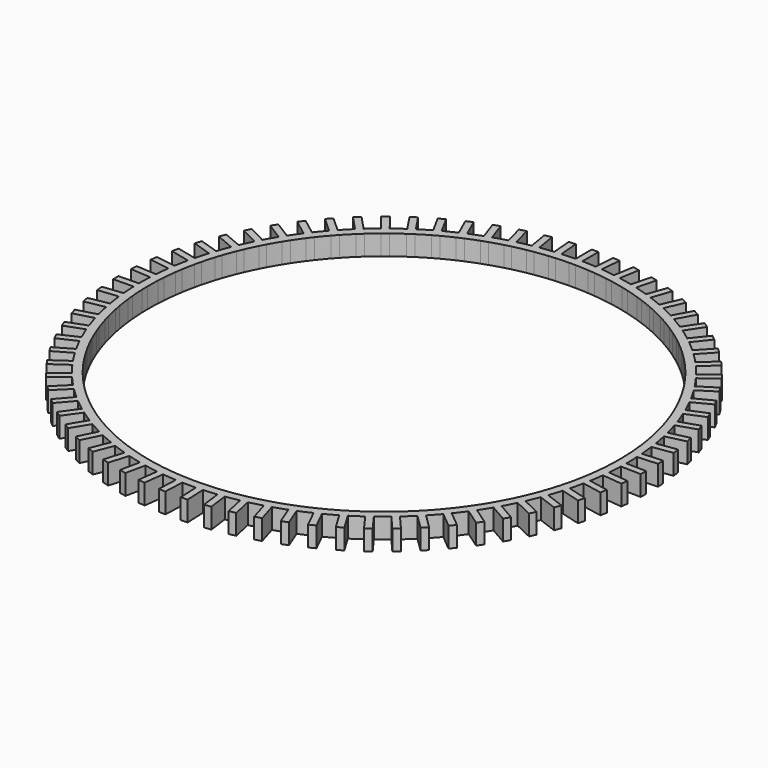
from build123d import *

# Parameters (mm, degrees)
F1_DEPTH = 3


# Not quite as in the source:
# - a feature names something its author has since deleted; it is built from what else it names


with BuildPart() as f1:
    # F0 (on Top) → F1 (new body)
    with BuildSketch(Plane.XY):
        with BuildLine():
            Line((31.2456081164, 15.7706047265), (32.3534717449, 16.349781835))
            ThreePointArc((32.3534717449, 16.349781835), (32.1248797471, 16.7944812731), (31.8901757098, 17.2359854142))
            Line((31.8901757098, 17.2359854142), (30.7823120813, 16.6568083057))
            ThreePointArc((30.7823120813, 16.6568083057), (31.0171252731, 16.2153612292), (31.2456081164, 15.7706047265))
        make_face()
        with BuildLine():
            ThreePointArc((23.3057460851, -27.7651706174), (23.6864968946, -27.4410707674), (24.0627411408, -27.1117500134))
            Line((24.0627411408, -27.1117500134), (23.2458849034, -26.1654129541))
            ThreePointArc((23.2458849034, -26.1654129541), (22.8697211397, -26.4948269478), (22.4888898477, -26.8188335581))
            Line((22.4888898477, -26.8188335581), (23.3057460851, -27.7651706174))
        make_face()
        with BuildLine():
            ThreePointArc((-21.7096969507, -29.0301835735), (-21.3072153956, -29.3268660461), (-20.9006799563, -29.6179688258))
            Line((-20.9006799563, -29.6179688258), (-20.1658759929, -28.6065979354))
            ThreePointArc((-20.1658759929, -28.6065979354), (-20.5724838302, -28.3155948031), (-20.9748929873, -28.0188126831))
            Line((-20.9748929873, -28.0188126831), (-21.7096969507, -29.0301835735))
        make_face()
        with BuildLine():
            Line((-32.068159976, 14.0225930468), (-33.2206024622, 14.5070352605))
            ThreePointArc((-33.2206024622, 14.5070352605), (-33.4175392451, 14.0474400089), (-33.6081180486, 13.5851721089))
            Line((-33.6081180486, 13.5851721089), (-32.4556755624, 13.1007298952))
            ThreePointArc((-32.4556755624, 13.1007298952), (-32.2652103056, 13.5630455258), (-32.068159976, 14.0225930468))
        make_face()
        with BuildLine():
            Line((-19.9048779878, -33.832060716), (-18.3490105747, -31.2630182633))
            ThreePointArc((-18.3490105747, -31.2630182633), (-18.7784790898, -31.0069544308), (-19.2043748349, -30.7449912539))
            Line((-19.2043748349, -30.7449912539), (-20.760242248, -33.3140337066))
            Line((-20.760242248, -33.3140337066), (-19.9048779878, -33.832060716))
        make_face()
        with BuildLine():
            ThreePointArc((30.3360622879, 19.8440375142), (30.6068872994, 19.423721318), (30.8718890828, 18.9997095887))
            Line((30.8718890828, 18.9997095887), (33.4077844734, 20.6090377402))
            Line((33.4077844734, 20.6090377402), (32.8719576785, 21.4533656657))
            Line((32.8719576785, 21.4533656657), (30.3360622879, 19.8440375142))
        make_face()
        with BuildLine():
            Line((28.3928843458, -27.1045497753), (26.2470024909, -25.0031470068))
            ThreePointArc((26.2470024909, -25.0031470068), (25.8996346367, -25.3627960936), (25.5473391503, -25.7176196865))
            Line((25.5473391503, -25.7176196865), (27.6932210053, -27.819022455))
            Line((27.6932210053, -27.819022455), (28.3928843458, -27.1045497753))
        make_face()
        with BuildLine():
            ThreePointArc((-12.8783573365, -33.8852536115), (-11.9214159443, -34.2336434211), (-10.9550656792, -34.5550146283))
            Line((-10.9550656792, -34.5550146283), (-10.5937403327, -33.3582473425))
            ThreePointArc((-10.5937403327, -33.3582473425), (-11.5103326359, -33.0531729583), (-12.4181563034, -32.7229184827))
            Line((-12.4181563034, -32.7229184827), (-12.8783573365, -33.8852536115))
        make_face()
        with BuildLine():
            Line((-34.6940398722, 4.6177480815), (-35.930752138, 4.8003698604))
            ThreePointArc((-35.930752138, 4.8003698604), (-36.0514187071, 3.7891567935), (-36.1436320106, 2.7749531678))
            Line((-36.1436320106, 2.7749531678), (-34.8959756722, 2.6964572844))
            ThreePointArc((-34.8959756722, 2.6964572844), (-34.8082663379, 3.6584962144), (-34.6940398722, 4.6177480815))
        make_face()
        with BuildLine():
            Line((25.6728493644, 23.7887537612), (26.6018719301, 24.6252494366))
            ThreePointArc((26.6018719301, 24.6252494366), (25.8996346367, 25.3627960936), (25.1769562841, 26.0803253866))
            Line((25.1769562841, 26.0803253866), (24.3211880854, 25.1690248146))
            ThreePointArc((24.3211880854, 25.1690248146), (25.0065437871, 24.488216918), (25.6728493644, 23.7887537612))
        make_face()
        with BuildLine():
            ThreePointArc((30.0491839313, -20.2758241526), (30.6068872994, -19.423721318), (31.1404344506, -18.5562884819))
            Line((31.1404344506, -18.5562884819), (30.0577960268, -17.9312268965))
            ThreePointArc((30.0577960268, -17.9312268965), (29.5514773926, -18.7539378243), (29.0226462781, -19.5623618976))
            Line((29.0226462781, -19.5623618976), (30.0491839313, -20.2758241526))
        make_face()
        with BuildLine():
            ThreePointArc((33.2206024622, 14.5070352605), (33.4175392451, 14.0474400089), (33.6081180486, 13.5851721089))
            Line((33.6081180486, 13.5851721089), (36.3768864931, 14.7490551925))
            Line((36.3768864931, 14.7490551925), (35.9893709066, 15.670918344))
            Line((35.9893709066, 15.670918344), (33.2206024622, 14.5070352605))
        make_face()
        with BuildLine():
            Line((23.4750796497, -31.4600244031), (21.7096969507, -29.0301835735))
            ThreePointArc((21.7096969507, -29.0301835735), (21.3072153956, -29.3268660461), (20.9006799563, -29.6179688258))
            Line((20.9006799563, -29.6179688258), (22.6660626553, -32.0478096554))
            Line((22.6660626553, -32.0478096554), (23.4750796497, -31.4600244031))
        make_face()
        with BuildLine():
            Line((-33.4380897638, 10.3389628565), (-34.6270275517, 10.7252721614))
            ThreePointArc((-34.6270275517, 10.7252721614), (-34.9146430464, 9.7483434973), (-35.1747024658, 8.7637210387))
            Line((-35.1747024658, 8.7637210387), (-33.9576089206, 8.4782543249))
            ThreePointArc((-33.9576089206, 8.4782543249), (-33.7106898379, 9.4121937215), (-33.4380897638, 10.3389628565))
        make_face()
        with BuildLine():
            ThreePointArc((26.2470024909, -25.0031470068), (26.9389999236, -24.2559844805), (27.6097359871, -23.4896781315))
            Line((27.6097359871, -23.4896781315), (26.6464995289, -22.6928196322))
            ThreePointArc((26.6464995289, -22.6928196322), (26.0100688917, -23.4195712226), (25.3538236391, -24.128481653))
            Line((25.3538236391, -24.128481653), (26.2470024909, -25.0031470068))
        make_face()
        with BuildLine():
            ThreePointArc((-18.3490105747, -31.2630182633), (-17.4635706862, -31.7661171516), (-16.5643478279, -32.2441449109))
            Line((-16.5643478279, -32.2441449109), (-16.0084990878, -31.124394885))
            ThreePointArc((-16.0084990878, -31.124394885), (-16.8613785936, -30.6707338015), (-17.7014130071, -30.1937075821))
            Line((-17.7014130071, -30.1937075821), (-18.3490105747, -31.2630182633))
        make_face()
        with BuildLine():
            ThreePointArc((31.8901757098, 17.2359854142), (32.1248797471, 16.7944812731), (32.3534717449, 16.349781835))
            Line((32.3534717449, 16.349781835), (35.0151385024, 17.7412675888))
            Line((35.0151385024, 17.7412675888), (34.5518424673, 18.6274711681))
            Line((34.5518424673, 18.6274711681), (31.8901757098, 17.2359854142))
        make_face()
        with BuildLine():
            Line((-22.6660626553, -32.0478096554), (-20.9006799563, -29.6179688258))
            ThreePointArc((-20.9006799563, -29.6179688258), (-21.3072153956, -29.3268660461), (-21.7096969507, -29.0301835735))
            Line((-21.7096969507, -29.0301835735), (-23.4750796497, -31.4600244031))
            Line((-23.4750796497, -31.4600244031), (-22.6660626553, -32.0478096554))
        make_face()
        with BuildLine():
            Line((-34.1859597907, 7.504675422), (-35.4030533359, 7.7901421358))
            ThreePointArc((-35.4030533359, 7.7901421358), (-35.6079128389, 6.7925726537), (-35.7846691095, 5.7896421933))
            Line((-35.7846691095, 5.7896421933), (-34.5479568437, 5.6070204144))
            ThreePointArc((-34.5479568437, 5.6070204144), (-34.3800537755, 6.5583460105), (-34.1859597907, 7.504675422))
        make_face()
        with BuildLine():
            Line((27.5734026786, 21.5570745865), (28.5691631854, 22.3128979491))
            ThreePointArc((28.5691631854, 22.3128979491), (27.9311050506, 23.1066196284), (27.2710025365, 23.8821046111))
            Line((27.2710025365, 23.8821046111), (26.3419799708, 23.0456089357))
            ThreePointArc((26.3419799708, 23.0456089357), (26.9679634972, 22.3098396412), (27.5734026786, 21.5570745865))
        make_face()
        with BuildLine():
            ThreePointArc((-15.6686360676, -32.6887800901), (-14.7442033115, -33.1160228395), (-13.8081338224, -33.5171290588))
            Line((-13.8081338224, -33.5171290588), (-13.3479327893, -32.35479393))
            ThreePointArc((-13.3479327893, -32.35479393), (-14.2357825077, -31.9740910175), (-15.1127873275, -31.5690300642))
            Line((-15.1127873275, -31.5690300642), (-15.6686360676, -32.6887800901))
        make_face()
        with BuildLine():
            ThreePointArc((20.9006799563, -29.6179688258), (21.3072153956, -29.3268660461), (21.7096969507, -29.0301835735))
            Line((21.7096969507, -29.0301835735), (20.9748929873, -28.0188126831))
            ThreePointArc((20.9748929873, -28.0188126831), (20.5724838302, -28.3155948031), (20.1658759929, -28.6065979354))
            Line((20.1658759929, -28.6065979354), (20.9006799563, -29.6179688258))
        make_face()
        with BuildLine():
            ThreePointArc((-24.0627411408, -27.1117500134), (-23.6864968946, -27.4410707674), (-23.3057460851, -27.7651706174))
            Line((-23.3057460851, -27.7651706174), (-22.4888898477, -26.8188335581))
            ThreePointArc((-22.4888898477, -26.8188335581), (-22.8697211397, -26.4948269478), (-23.2458849034, -26.1654129541))
            Line((-23.2458849034, -26.1654129541), (-24.0627411408, -27.1117500134))
        make_face()
        with BuildLine():
            Line((-30.7823120813, 16.6568083057), (-31.8901757098, 17.2359854142))
            ThreePointArc((-31.8901757098, 17.2359854142), (-32.1248797471, 16.7944812731), (-32.3534717449, 16.349781835))
            Line((-32.3534717449, 16.349781835), (-31.2456081164, 15.7706047265))
            ThreePointArc((-31.2456081164, 15.7706047265), (-31.0171252731, 16.2153612292), (-30.7823120813, 16.6568083057))
        make_face()
        with BuildLine():
            ThreePointArc((-35.4030533359, 7.7901421358), (-35.2922352292, 8.2777190415), (-35.1747024658, 8.7637210387))
            Line((-35.1747024658, 8.7637210387), (-38.0987965027, 9.4495611033))
            Line((-38.0987965027, 9.4495611033), (-38.3271473728, 8.4759822004))
            Line((-38.3271473728, 8.4759822004), (-35.4030533359, 7.7901421358))
        make_face()
        with BuildLine():
            ThreePointArc((28.5691631854, 22.3128979491), (28.8742095284, 21.9167179138), (29.1737623003, 21.516368031))
            Line((29.1737623003, 21.516368031), (31.5660988399, 23.3322502993))
            Line((31.5660988399, 23.3322502993), (30.961499725, 24.1287802174))
            Line((30.961499725, 24.1287802174), (28.5691631854, 22.3128979491))
        make_face()
        with BuildLine():
            Line((-34.9587661917, 1.698430556), (-36.2064225301, 1.7769264394))
            ThreePointArc((-36.2064225301, 1.7769264394), (-36.242049776, 0.7591627208), (-36.2490733023, -0.2592001604))
            Line((-36.2490733023, -0.2592001604), (-34.9992243041, -0.233019556))
            ThreePointArc((-34.9992243041, -0.233019556), (-34.9923239216, 0.7329846959), (-34.9587661917, 1.698430556))
        make_face()
        with BuildLine():
            Line((-6.3293085205, 34.42295533), (-6.537789995, 35.6555718224))
            ThreePointArc((-6.537789995, 35.6555718224), (-7.5367987921, 35.4578505266), (-8.529859237, 35.2321444337))
            Line((-8.529859237, 35.2321444337), (-8.2189662467, 34.021296181))
            ThreePointArc((-8.2189662467, 34.021296181), (-7.2769091786, 34.2351660257), (-6.3293085205, 34.42295533))
        make_face()
        with BuildLine():
            Line((23.592219458, 25.8535719205), (24.4479876567, 26.7648724925))
            ThreePointArc((24.4479876567, 26.7648724925), (23.6864968946, 27.4410707674), (22.906311773, 28.0956114181))
            Line((22.906311773, 28.0956114181), (22.1298005403, 27.1158980682))
            ThreePointArc((22.1298005403, 27.1158980682), (22.8697211397, 26.4948269478), (23.592219458, 25.8535719205))
        make_face()
        with BuildLine():
            ThreePointArc((31.6404344506, -17.6902630782), (32.1248797471, -16.7944812731), (32.5839707644, -15.8854445712))
            Line((32.5839707644, -15.8854445712), (31.4528255005, -15.3531680131))
            ThreePointArc((31.4528255005, -15.3531680131), (31.0171252731, -16.2153612292), (30.5577960268, -17.0652014927))
            Line((30.5577960268, -17.0652014927), (31.6404344506, -17.6902630782))
        make_face()
        with BuildLine():
            ThreePointArc((-9.9977461817, -34.8440464253), (-9.0150084097, -35.1111395909), (-8.0251556215, -35.350521598))
            Line((-8.0251556215, -35.350521598), (-7.7652403993, -34.1277166177))
            ThreePointArc((-7.7652403993, -34.1277166177), (-8.7041460508, -33.9004106395), (-9.6364208352, -33.6472791394))
            Line((-9.6364208352, -33.6472791394), (-9.9977461817, -34.8440464253))
        make_face()
        with BuildLine():
            ThreePointArc((-35.930752138, 4.8003698604), (-35.8611220699, 5.2955097854), (-35.7846691095, 5.7896421933))
            Line((-35.7846691095, 5.7896421933), (-38.7558975545, 6.2283950376))
            Line((-38.7558975545, 6.2283950376), (-38.9019805831, 5.2391227046))
            Line((-38.9019805831, 5.2391227046), (-35.930752138, 4.8003698604))
        make_face()
        with BuildLine():
            ThreePointArc((26.6018719301, 24.6252494366), (26.9389999236, 24.2559844805), (27.2710025365, 23.8821046111))
            Line((27.2710025365, 23.8821046111), (29.5029997032, 25.8918038868))
            Line((29.5029997032, 25.8918038868), (28.8338690968, 26.6349487123))
            Line((28.8338690968, 26.6349487123), (26.6018719301, 24.6252494366))
        make_face()
        with BuildLine():
            Line((32.5154632423, -21.989932927), (30.0491839313, -20.2758241526))
            ThreePointArc((30.0491839313, -20.2758241526), (29.7666588311, -20.6883668286), (29.4784703636, -21.0969733617))
            Line((29.4784703636, -21.0969733617), (31.9447496747, -22.8110821362))
            Line((31.9447496747, -22.8110821362), (32.5154632423, -21.989932927))
        make_face()
        with BuildLine():
            ThreePointArc((-36.2281308824, -1.2589808438), (-36.1784689055, -2.2761563329), (-36.1002533898, -3.2915353856))
            Line((-36.1002533898, -3.2915353856), (-34.8569785244, -3.1608619317))
            ThreePointArc((-34.8569785244, -3.1608619317), (-34.930935495, -2.1976681835), (-34.9782818842, -1.2328002395))
            Line((-34.9782818842, -1.2328002395), (-36.2281308824, -1.2589808438))
        make_face()
        with BuildLine():
            Line((-9.1875494078, 33.7726062938), (-9.4984423982, 34.9834545465))
            ThreePointArc((-9.4984423982, 34.9834545465), (-10.4774026392, 34.7028317855), (-11.4480936823, 34.3948201193))
            Line((-11.4480936823, 34.3948201193), (-11.0369698671, 33.2142333368))
            ThreePointArc((-11.0369698671, 33.2142333368), (-10.1161128931, 33.5061824136), (-9.1875494078, 33.7726062938))
        make_face()
        with BuildLine():
            Line((21.346107083, 27.7370458485), (22.1226183156, 28.7167591984))
            ThreePointArc((22.1226183156, 28.7167591984), (21.3072153956, 29.3268660461), (20.4749959429, 29.9138269223))
            Line((20.4749959429, 29.9138269223), (19.7831883446, 28.8725727797))
            ThreePointArc((19.7831883446, 28.8725727797), (20.5724838302, 28.3155948031), (21.346107083, 27.7370458485))
        make_face()
        with BuildLine():
            ThreePointArc((-7.0470080208, -35.5584332888), (-6.0453670685, -35.7423563438), (-5.0389548632, -35.898070058))
            Line((-5.0389548632, -35.898070058), (-4.8822728839, -34.6578044816))
            ThreePointArc((-4.8822728839, -34.6578044816), (-5.8369061351, -34.5098612975), (-6.7870927986, -34.3356283086))
            Line((-6.7870927986, -34.3356283086), (-7.0470080208, -35.5584332888))
        make_face()
        with BuildLine():
            ThreePointArc((27.6097359871, -23.4896781315), (27.9311050506, -23.1066196284), (28.2471599769, -22.7191648887))
            Line((28.2471599769, -22.7191648887), (27.2839235186, -21.9223063894))
            ThreePointArc((27.2839235186, -21.9223063894), (26.9679634972, -22.3098396412), (26.6464995289, -22.6928196322))
            Line((26.6464995289, -22.6928196322), (27.6097359871, -23.4896781315))
        make_face()
        with BuildLine():
            ThreePointArc((-36.2064225301, 1.7769264394), (-36.1784689055, 2.2761563329), (-36.1436320106, 2.7749531678))
            Line((-36.1436320106, 2.7749531678), (-39.141153831, 2.9635412557))
            Line((-39.141153831, 2.9635412557), (-39.2039443506, 1.9655145273))
            Line((-39.2039443506, 1.9655145273), (-36.2064225301, 1.7769264394))
        make_face()
        with BuildLine():
            ThreePointArc((24.4479876567, 26.7648724925), (24.8148325899, 26.425112744), (25.1769562841, 26.0803253866))
            Line((25.1769562841, 26.0803253866), (27.2329582214, 28.2697450733))
            Line((27.2329582214, 28.2697450733), (26.503989594, 28.9542921793))
            Line((26.503989594, 28.9542921793), (24.4479876567, 26.7648724925))
        make_face()
        with BuildLine():
            Line((-10.8658382813, -37.7193061766), (-9.9977461817, -34.8440464253))
            ThreePointArc((-9.9977461817, -34.8440464253), (-10.4774026392, -34.7028317855), (-10.9550656792, -34.5550146283))
            Line((-10.9550656792, -34.5550146283), (-11.8231577788, -37.4302743797))
            Line((-11.8231577788, -37.4302743797), (-10.8658382813, -37.7193061766))
        make_face()
        with BuildLine():
            Line((-11.9813462373, 32.8853666901), (-12.3924700525, 34.0659534726))
            ThreePointArc((-12.3924700525, 34.0659534726), (-13.3445150348, 33.7043976134), (-14.2860279758, 33.3162408545))
            Line((-14.2860279758, 33.3162408545), (-13.7775570738, 32.1741965102))
            ThreePointArc((-13.7775570738, 32.1741965102), (-12.884359344, 32.5421770061), (-11.9813462373, 32.8853666901))
        make_face()
        with BuildLine():
            Line((18.9502671039, 29.425964329), (19.6420747022, 30.4672184715))
            ThreePointArc((19.6420747022, 30.4672184715), (18.7784790898, 31.0069544308), (17.9000627276, 31.5222184236))
            Line((17.9000627276, 31.5222184236), (17.297811297, 30.4267271381))
            ThreePointArc((17.297811297, 30.4267271381), (18.1309453281, 29.9377491056), (18.9502671039, 29.425964329))
        make_face()
        with BuildLine():
            ThreePointArc((34.1475259821, -12.1658936909), (34.4757987157, -11.2018660461), (34.7768617279, -10.2289974269))
            Line((34.7768617279, -10.2289974269), (33.5727898858, -9.892814528))
            ThreePointArc((33.5727898858, -9.892814528), (33.2869780703, -10.8155948031), (32.9758080494, -11.7301356978))
            Line((32.9758080494, -11.7301356978), (34.1475259821, -12.1658936909))
        make_face()
        with BuildLine():
            ThreePointArc((-4.0468401619, -36.0234032915), (-3.0333218208, -36.1228661478), (-2.0174094571, -36.1938193492))
            Line((-2.0174094571, -36.1938193492), (-1.965059732, -34.9447927487))
            ThreePointArc((-1.965059732, -34.9447927487), (-2.9287245166, -34.8772500737), (-3.8901581826, -34.7831377152))
            Line((-3.8901581826, -34.7831377152), (-4.0468401619, -36.0234032915))
        make_face()
        with BuildLine():
            ThreePointArc((29.4784703636, -21.0969733617), (29.7666588311, -20.6883668286), (30.0491839313, -20.2758241526))
            Line((30.0491839313, -20.2758241526), (29.0226462781, -19.5623618976))
            ThreePointArc((29.0226462781, -19.5623618976), (28.7402223197, -19.974974869), (28.4519327104, -20.3835111068))
            Line((28.4519327104, -20.3835111068), (29.4784703636, -21.0969733617))
        make_face()
        with BuildLine():
            Line((-34.5479568437, 5.6070204144), (-35.7846691095, 5.7896421933))
            ThreePointArc((-35.7846691095, 5.7896421933), (-35.8611220699, 5.2955097854), (-35.930752138, 4.8003698604))
            Line((-35.930752138, 4.8003698604), (-34.6940398722, 4.6177480815))
            ThreePointArc((-34.6940398722, 4.6177480815), (-34.6245316537, 5.1129059997), (-34.5479568437, 5.6070204144))
        make_face()
        with BuildLine():
            Line((-2.4301792223, 34.9155299107), (-2.5347868332, 36.1612687237))
            ThreePointArc((-2.5347868332, 36.1612687237), (-3.0333218208, 36.1228661478), (-3.5312796924, 36.0775908804))
            Line((-3.5312796924, 36.0775908804), (-3.4266720816, 34.8318520674))
            ThreePointArc((-3.4266720816, 34.8318520674), (-2.9287245166, 34.8772500737), (-2.4301792223, 34.9155299107))
        make_face()
        with BuildLine():
            Line((35.7273514551, -16.2594236677), (33.009750056, -14.9806175187))
            ThreePointArc((33.009750056, -14.9806175187), (32.7999806519, -15.4344993192), (32.5839707644, -15.8854445712))
            Line((32.5839707644, -15.8854445712), (35.3015721635, -17.1642507202))
            Line((35.3015721635, -17.1642507202), (35.7273514551, -16.2594236677))
        make_face()
        with BuildLine():
            Line((-7.6714600642, -38.4962491742), (-7.0470080208, -35.5584332888))
            ThreePointArc((-7.0470080208, -35.5584332888), (-7.5367987921, -35.4578505266), (-8.0251556215, -35.350521598))
            Line((-8.0251556215, -35.350521598), (-8.649607665, -38.2883374834))
            Line((-8.649607665, -38.2883374834), (-7.6714600642, -38.4962491742))
        make_face()
        with BuildLine():
            Line((-14.6911025315, 31.7674598671), (-15.1995734335, 32.9095042114))
            ThreePointArc((-15.1995734335, 32.9095042114), (-16.1180252455, 32.4695513087), (-17.0237560476, 32.0039720977))
            Line((-17.0237560476, 32.0039720977), (-16.4215046169, 30.9084808122))
            ThreePointArc((-16.4215046169, 30.9084808122), (-15.5622312715, 31.3499116084), (-14.6911025315, 31.7674598671))
        make_face()
        with BuildLine():
            Line((16.4215046169, 30.9084808122), (17.0237560476, 32.0039720977))
            ThreePointArc((17.0237560476, 32.0039720977), (16.1180252455, 32.4695513087), (15.1995734335, 32.9095042114))
            Line((15.1995734335, 32.9095042114), (14.6911025315, 31.7674598671))
            ThreePointArc((14.6911025315, 31.7674598671), (15.5622312715, 31.3499116084), (16.4215046169, 30.9084808122))
        make_face()
        with BuildLine():
            ThreePointArc((-1.018286627, -36.2356950029), (0, -36.25), (1.018286627, -36.2356950029))
            Line((1.018286627, -36.2356950029), (0.9659369019, -34.9866684024))
            ThreePointArc((0.9659369019, -34.9866684024), (0, -35), (-0.9659369019, -34.9866684024))
            Line((-0.9659369019, -34.9866684024), (-1.018286627, -36.2356950029))
        make_face()
        with BuildLine():
            Line((-5.3433124835, 34.5897240767), (-5.5517939579, 35.8223405691))
            ThreePointArc((-5.5517939579, 35.8223405691), (-6.0453670685, 35.7423563438), (-6.537789995, 35.6555718224))
            Line((-6.537789995, 35.6555718224), (-6.3293085205, 34.42295533))
            ThreePointArc((-6.3293085205, 34.42295533), (-5.8369061351, 34.5098612975), (-5.3433124835, 34.5897240767))
        make_face()
        with BuildLine():
            Line((-38.9827201616, -4.6000031309), (-35.9957249265, -4.286057281))
            ThreePointArc((-35.9957249265, -4.286057281), (-36.0514187071, -3.7891567935), (-36.1002533898, -3.2915353856))
            Line((-36.1002533898, -3.2915353856), (-39.0872486248, -3.6054812356))
            Line((-39.0872486248, -3.6054812356), (-38.9827201616, -4.6000031309))
        make_face()
        with BuildLine():
            Line((36.9626041112, -13.2128118626), (34.1475259821, -12.1658936909))
            ThreePointArc((34.1475259821, -12.1658936909), (33.9764721191, -12.6357367154), (33.7989539348, -13.1031756804))
            Line((33.7989539348, -13.1031756804), (36.6140320639, -14.1500938521))
            Line((36.6140320639, -14.1500938521), (36.9626041112, -13.2128118626))
        make_face()
        with BuildLine():
            Line((-4.4232720667, -39.0031686434), (-4.0468401619, -36.0234032915))
            ThreePointArc((-4.0468401619, -36.0234032915), (-4.5433297167, -35.9641579226), (-5.0389548632, -35.898070058))
            Line((-5.0389548632, -35.898070058), (-5.4153867681, -38.8778354098))
            Line((-5.4153867681, -38.8778354098), (-4.4232720667, -39.0031686434))
        make_face()
        with BuildLine():
            ThreePointArc((-34.7768617279, -10.2289974269), (-34.4757987157, -11.2018660461), (-34.1475259821, -12.1658936909))
            Line((-34.1475259821, -12.1658936909), (-32.9758080494, -11.7301356978))
            ThreePointArc((-32.9758080494, -11.7301356978), (-33.2869780703, -10.8155948031), (-33.5727898858, -9.892814528))
            Line((-33.5727898858, -9.892814528), (-34.7768617279, -10.2289974269))
        make_face()
        with BuildLine():
            Line((13.7775570738, 32.1741965102), (14.2860279758, 33.3162408545))
            ThreePointArc((14.2860279758, 33.3162408545), (13.3445150348, 33.7043976134), (12.3924700525, 34.0659534726))
            Line((12.3924700525, 34.0659534726), (11.9813462373, 32.8853666901))
            ThreePointArc((11.9813462373, 32.8853666901), (12.884359344, 32.5421770061), (13.7775570738, 32.1741965102))
        make_face()
        with BuildLine():
            ThreePointArc((35.6982161377, -6.3007828552), (35.8611220699, -5.2955097854), (35.9957249265, -4.286057281))
            Line((35.9957249265, -4.286057281), (34.7524500611, -4.1553838271))
            ThreePointArc((34.7524500611, -4.1553838271), (34.6245316537, -5.1129059997), (34.470236085, -6.066533132))
            Line((34.470236085, -6.066533132), (35.6982161377, -6.3007828552))
        make_face()
        with BuildLine():
            ThreePointArc((2.0174094571, -36.1938193492), (3.0333218208, -36.1228661478), (4.0468401619, -36.0234032915))
            Line((4.0468401619, -36.0234032915), (3.8901581826, -34.7831377152))
            ThreePointArc((3.8901581826, -34.7831377152), (2.9287245166, -34.8772500737), (1.965059732, -34.9447927487))
            Line((1.965059732, -34.9447927487), (2.0174094571, -36.1938193492))
        make_face()
        with BuildLine():
            ThreePointArc((32.5839707644, -15.8854445712), (32.7999806519, -15.4344993192), (33.009750056, -14.9806175187))
            Line((33.009750056, -14.9806175187), (31.878604792, -14.4483409606))
            ThreePointArc((31.878604792, -14.4483409606), (31.6689468363, -14.9022752048), (31.4528255005, -15.3531680131))
            Line((31.4528255005, -15.3531680131), (32.5839707644, -15.8854445712))
        make_face()
        with BuildLine():
            Line((-38.4610839338, -7.8458602229), (-35.5108348231, -7.2830701059))
            ThreePointArc((-35.5108348231, -7.2830701059), (-35.6079128389, -6.7925726537), (-35.6982161377, -6.3007828552))
            Line((-35.6982161377, -6.3007828552), (-38.6484652484, -6.8635729721))
            Line((-38.6484652484, -6.8635729721), (-38.4610839338, -7.8458602229))
        make_face()
        with BuildLine():
            ThreePointArc((17.0237560476, 32.0039720977), (17.4635706862, 31.7661171516), (17.9000627276, 31.5222184236))
            Line((17.9000627276, 31.5222184236), (19.3469850485, 34.1541603547))
            Line((19.3469850485, 34.1541603547), (18.4706783685, 34.6359140288))
            Line((18.4706783685, 34.6359140288), (17.0237560476, 32.0039720977))
        make_face()
        with BuildLine():
            Line((-19.7831883446, 28.8725727797), (-20.4749959429, 29.9138269223))
            ThreePointArc((-20.4749959429, 29.9138269223), (-21.3072153956, 29.3268660461), (-22.1226183156, 28.7167591984))
            Line((-22.1226183156, 28.7167591984), (-21.346107083, 27.7370458485))
            ThreePointArc((-21.346107083, 27.7370458485), (-20.5724838302, 28.3155948031), (-19.7831883446, 28.8725727797))
        make_face()
        with BuildLine():
            Line((11.0369698671, 33.2142333368), (11.4480936823, 34.3948201193))
            ThreePointArc((11.4480936823, 34.3948201193), (10.4774026392, 34.7028317855), (9.4984423982, 34.9834545465))
            Line((9.4984423982, 34.9834545465), (9.1875494078, 33.7726062938))
            ThreePointArc((9.1875494078, 33.7726062938), (10.1161128931, 33.5061824136), (11.0369698671, 33.2142333368))
        make_face()
        with BuildLine():
            ThreePointArc((36.1002533898, -3.2915353856), (36.1784689055, -2.2761563329), (36.2281308824, -1.2589808438))
            Line((36.2281308824, -1.2589808438), (34.9782818842, -1.2328002395))
            ThreePointArc((34.9782818842, -1.2328002395), (34.930935495, -2.1976681835), (34.8569785244, -3.1608619317))
            Line((34.8569785244, -3.1608619317), (36.1002533898, -3.2915353856))
        make_face()
        with BuildLine():
            ThreePointArc((-5.0389548632, -35.898070058), (-4.5433297167, -35.9641579226), (-4.0468401619, -36.0234032915))
            Line((-4.0468401619, -36.0234032915), (-3.8901581826, -34.7831377152))
            ThreePointArc((-3.8901581826, -34.7831377152), (-4.3866631748, -34.724014546), (-4.8822728839, -34.6578044816))
            Line((-4.8822728839, -34.6578044816), (-5.0389548632, -35.898070058))
        make_face()
        with BuildLine():
            Line((-11.0369698671, 33.2142333368), (-11.4480936823, 34.3948201193))
            ThreePointArc((-11.4480936823, 34.3948201193), (-11.9214159443, 34.2336434211), (-12.3924700525, 34.0659534726))
            Line((-12.3924700525, 34.0659534726), (-11.9813462373, 32.8853666901))
            ThreePointArc((-11.9813462373, 32.8853666901), (-11.5103326359, 33.0531729583), (-11.0369698671, 33.2142333368))
        make_face()
        with BuildLine():
            ThreePointArc((14.2860279758, 33.3162408545), (14.7442033115, 33.1160228395), (15.1995734335, 32.9095042114))
            Line((15.1995734335, 32.9095042114), (16.4211859695, 35.6532908909))
            Line((16.4211859695, 35.6532908909), (15.5076405119, 36.060027534))
            Line((15.5076405119, 36.060027534), (14.2860279758, 33.3162408545))
        make_face()
        with BuildLine():
            ThreePointArc((36.2490733023, -0.2592001604), (36.2497683248, -0.1296009085), (36.25, 0))
            ThreePointArc((36.25, 0), (36.239103995, 0.8887303538), (36.2064225301, 1.7769264394))
            Line((36.2064225301, 1.7769264394), (34.9587661917, 1.698430556))
            ThreePointArc((34.9587661917, 1.698430556), (34.9896900294, 0.8494655056), (35, 0))
            ThreePointArc((35, 0), (34.9998060755, -0.1165104236), (34.9992243041, -0.233019556))
            Line((34.9992243041, -0.233019556), (36.2490733023, -0.2592001604))
        make_face()
        with BuildLine():
            ThreePointArc((8.0251556215, -35.350521598), (9.0150084097, -35.1111395909), (9.9977461817, -34.8440464253))
            Line((9.9977461817, -34.8440464253), (9.6364208352, -33.6472791394))
            ThreePointArc((9.6364208352, -33.6472791394), (8.7041460508, -33.9004106395), (7.7652403993, -34.1277166177))
            Line((7.7652403993, -34.1277166177), (8.0251556215, -35.350521598))
        make_face()
        with BuildLine():
            ThreePointArc((-32.5839707644, -15.8854445712), (-32.1248797471, -16.7944812731), (-31.6404344506, -17.6902630782))
            Line((-31.6404344506, -17.6902630782), (-30.5577960268, -17.0652014927))
            ThreePointArc((-30.5577960268, -17.0652014927), (-31.0171252731, -16.2153612292), (-31.4528255004, -15.3531680131))
            Line((-31.4528255005, -15.3531680131), (-32.5839707644, -15.8854445712))
        make_face()
        with BuildLine():
            Line((-22.1298005403, 27.1158980682), (-22.906311773, 28.0956114181))
            ThreePointArc((-22.906311773, 28.0956114181), (-23.6864968946, 27.4410707674), (-24.4479876567, 26.7648724925))
            Line((-24.4479876567, 26.7648724925), (-23.592219458, 25.8535719205))
            ThreePointArc((-23.592219458, 25.8535719205), (-22.8697211397, 26.4948269478), (-22.1298005403, 27.1158980682))
        make_face()
        with BuildLine():
            ThreePointArc((-35.6982161377, -6.3007828552), (-35.6079128389, -6.7925726537), (-35.5108348231, -7.2830701059))
            Line((-35.5108348231, -7.2830701059), (-34.2828547705, -7.0488203827))
            ThreePointArc((-34.2828547705, -7.0488203827), (-34.3800537755, -6.5583460105), (-34.470236085, -6.066533132))
            Line((-34.470236085, -6.066533132), (-35.6982161377, -6.3007828552))
        make_face()
        with BuildLine():
            Line((-13.7775570738, 32.1741965102), (-14.2860279758, 33.3162408545))
            ThreePointArc((-14.2860279758, 33.3162408545), (-14.7442033115, 33.1160228395), (-15.1995734335, 32.9095042114))
            Line((-15.1995734335, 32.9095042114), (-14.6911025315, 31.7674598671))
            ThreePointArc((-14.6911025315, 31.7674598671), (-14.2357825077, 31.9740910175), (-13.7775570738, 32.1741965102))
        make_face()
        with BuildLine():
            ThreePointArc((34.7768617279, -10.2289974269), (34.9146430464, -9.7483434973), (35.0457815485, -9.2658348601))
            Line((35.0457815485, -9.2658348601), (33.8417097064, -8.9296519612))
            ThreePointArc((33.8417097064, -8.9296519612), (33.7106898379, -9.4121937215), (33.5727898858, -9.892814528))
            Line((33.5727898858, -9.892814528), (34.7768617279, -10.2289974269))
        make_face()
        with BuildLine():
            Line((38.6484652484, -6.8635729721), (35.6982161377, -6.3007828552))
            ThreePointArc((35.6982161377, -6.3007828552), (35.6079128389, -6.7925726537), (35.5108348231, -7.2830701059))
            Line((35.5108348231, -7.2830701059), (38.4610839338, -7.8458602229))
            Line((38.4610839338, -7.8458602229), (38.6484652484, -6.8635729721))
        make_face()
        with BuildLine():
            Line((-37.6696708365, -11.0366842425), (-34.7768617279, -10.2289974269))
            ThreePointArc((-34.7768617279, -10.2289974269), (-34.9146430464, -9.7483434973), (-35.0457815485, -9.2658348601))
            Line((-35.0457815485, -9.2658348601), (-37.9385906571, -10.0735216758))
            Line((-37.9385906571, -10.0735216758), (-37.6696708365, -11.0366842425))
        make_face()
        with BuildLine():
            Line((34.8959756722, 2.6964572844), (36.1436320106, 2.7749531678))
            ThreePointArc((36.1436320106, 2.7749531678), (36.0514187071, 3.7891567935), (35.930752138, 4.8003698604))
            Line((35.930752138, 4.8003698604), (34.6940398722, 4.6177480815))
            ThreePointArc((34.6940398722, 4.6177480815), (34.8082663379, 3.6584962144), (34.8959756722, 2.6964572844))
        make_face()
        with BuildLine():
            ThreePointArc((10.9550656792, -34.5550146283), (11.9214159443, -34.2336434211), (12.8783573365, -33.8852536115))
            Line((12.8783573365, -33.8852536115), (12.4181563034, -32.7229184827))
            ThreePointArc((12.4181563034, -32.7229184827), (11.5103326359, -33.0531729583), (10.5937403327, -33.3582473425))
            Line((10.5937403327, -33.3582473425), (10.9550656792, -34.5550146283))
        make_face()
        with BuildLine():
            ThreePointArc((-31.1404344506, -18.5562884819), (-30.6068872994, -19.423721318), (-30.0491839313, -20.2758241526))
            Line((-30.0491839313, -20.2758241526), (-29.0226462781, -19.5623618976))
            ThreePointArc((-29.0226462781, -19.5623618976), (-29.5514773926, -18.7539378243), (-30.0577960268, -17.9312268965))
            Line((-30.0577960268, -17.9312268965), (-31.1404344506, -18.5562884819))
        make_face()
        with BuildLine():
            ThreePointArc((-35.0457815485, -9.2658348601), (-34.9146430464, -9.7483434973), (-34.7768617279, -10.2289974269))
            Line((-34.7768617279, -10.2289974269), (-33.5727898858, -9.892814528))
            ThreePointArc((-33.5727898858, -9.892814528), (-33.7106898379, -9.4121937215), (-33.8417097064, -8.9296519612))
            Line((-33.8417097064, -8.9296519612), (-35.0457815485, -9.2658348601))
        make_face()
        with BuildLine():
            ThreePointArc((35.5108348231, -7.2830701059), (35.6079128389, -6.7925726537), (35.6982161377, -6.3007828552))
            Line((35.6982161377, -6.3007828552), (34.470236085, -6.066533132))
            ThreePointArc((34.470236085, -6.066533132), (34.3800537755, -6.5583460105), (34.2828547705, -7.0488203827))
            Line((34.2828547705, -7.0488203827), (35.5108348231, -7.2830701059))
        make_face()
        with BuildLine():
            Line((39.0872486248, -3.6054812356), (36.1002533898, -3.2915353856))
            ThreePointArc((36.1002533898, -3.2915353856), (36.0514187071, -3.7891567935), (35.9957249265, -4.286057281))
            Line((35.9957249265, -4.286057281), (38.9827201616, -4.6000031309))
            Line((38.9827201616, -4.6000031309), (39.0872486248, -3.6054812356))
        make_face()
        with BuildLine():
            Line((5.4153867681, -38.8778354098), (5.0389548632, -35.898070058))
            ThreePointArc((5.0389548632, -35.898070058), (4.5433297167, -35.9641579226), (4.0468401619, -36.0234032915))
            Line((4.0468401619, -36.0234032915), (4.4232720667, -39.0031686434))
            Line((4.4232720667, -39.0031686434), (5.4153867681, -38.8778354098))
        make_face()
        with BuildLine():
            Line((-36.6140320639, -14.1500938521), (-33.7989539348, -13.1031756804))
            ThreePointArc((-33.7989539348, -13.1031756804), (-33.9764721191, -12.6357367154), (-34.1475259821, -12.1658936909))
            Line((-34.1475259821, -12.1658936909), (-36.9626041112, -13.2128118626))
            Line((-36.9626041112, -13.2128118626), (-36.6140320639, -14.1500938521))
        make_face()
        with BuildLine():
            Line((2.4301792223, 34.9155299107), (2.5347868332, 36.1612687237))
            ThreePointArc((2.5347868332, 36.1612687237), (1.5179924477, 36.2182025911), (0.5, 36.2465515601))
            Line((0.5, 36.2465515601), (0.5, 34.9964283892))
            ThreePointArc((0.5, 34.9964283892), (1.4656478805, 34.9692990535), (2.4301792223, 34.9155299107))
        make_face()
        with BuildLine():
            Line((11.9813462373, 32.8853666901), (12.3924700525, 34.0659534726))
            ThreePointArc((12.3924700525, 34.0659534726), (11.9214159443, 34.2336434211), (11.4480936823, 34.3948201193))
            Line((11.4480936823, 34.3948201193), (11.0369698671, 33.2142333368))
            ThreePointArc((11.0369698671, 33.2142333368), (11.5103326359, 33.0531729583), (11.9813462373, 32.8853666901))
        make_face()
        with BuildLine():
            ThreePointArc((4.0468401619, -36.0234032915), (4.5433297167, -35.9641579226), (5.0389548632, -35.898070058))
            Line((5.0389548632, -35.898070058), (4.8822728839, -34.6578044816))
            ThreePointArc((4.8822728839, -34.6578044816), (4.3866631748, -34.724014546), (3.8901581826, -34.7831377152))
            Line((3.8901581826, -34.7831377152), (4.0468401619, -36.0234032915))
        make_face()
        with BuildLine():
            Line((8.649607665, -38.2883374834), (8.0251556215, -35.350521598))
            ThreePointArc((8.0251556215, -35.350521598), (7.5367987921, -35.4578505266), (7.0470080208, -35.5584332888))
            Line((7.0470080208, -35.5584332888), (7.6714600642, -38.4962491742))
            Line((7.6714600642, -38.4962491742), (8.649607665, -38.2883374834))
        make_face()
        with BuildLine():
            Line((-35.3015721635, -17.1642507202), (-32.5839707644, -15.8854445712))
            ThreePointArc((-32.5839707644, -15.8854445712), (-32.7999806519, -15.4344993192), (-33.009750056, -14.9806175187))
            Line((-33.009750056, -14.9806175187), (-35.7273514551, -16.2594236677))
            Line((-35.7273514551, -16.2594236677), (-35.3015721635, -17.1642507202))
        make_face()
        with BuildLine():
            ThreePointArc((8.529859237, 35.2321444337), (9.0150084097, 35.1111395909), (9.4984423982, 34.9834545465))
            Line((9.4984423982, 34.9834545465), (10.2453696518, 37.8925441307))
            Line((10.2453696518, 37.8925441307), (9.2767864907, 38.1412340179))
            Line((9.2767864907, 38.1412340179), (8.529859237, 35.2321444337))
        make_face()
        with BuildLine():
            Line((34.5479568437, 5.6070204144), (35.7846691095, 5.7896421933))
            ThreePointArc((35.7846691095, 5.7896421933), (35.6079128389, 6.7925726537), (35.4030533359, 7.7901421358))
            Line((35.4030533359, 7.7901421358), (34.1859597907, 7.504675422))
            ThreePointArc((34.1859597907, 7.504675422), (34.3800537755, 6.5583460105), (34.5479568437, 5.6070204144))
        make_face()
        with BuildLine():
            ThreePointArc((13.8081338224, -33.5171290588), (14.7442033115, -33.1160228395), (15.6686360676, -32.6887800901))
            Line((15.6686360676, -32.6887800901), (15.1127873275, -31.5690300642))
            ThreePointArc((15.1127873275, -31.5690300642), (14.2357825077, -31.9740910175), (13.3479327893, -32.35479393))
            Line((13.3479327893, -32.35479393), (13.8081338224, -33.5171290588))
        make_face()
        with BuildLine():
            ThreePointArc((36.2281308824, -1.2589808438), (36.242049776, -0.7591627208), (36.2490733023, -0.2592001604))
            Line((36.2490733023, -0.2592001604), (34.9992243041, -0.233019556))
            ThreePointArc((34.9992243041, -0.233019556), (34.9923239216, -0.7329846959), (34.9782818842, -1.2328002395))
            Line((34.9782818842, -1.2328002395), (36.2281308824, -1.2589808438))
        make_face()
        with BuildLine():
            ThreePointArc((36.1436320106, 2.7749531678), (36.1784689055, 2.2761563329), (36.2064225301, 1.7769264394))
            Line((36.2064225301, 1.7769264394), (39.2039443506, 1.9655145273))
            Line((39.2039443506, 1.9655145273), (39.141153831, 2.9635412557))
            Line((39.141153831, 2.9635412557), (36.1436320106, 2.7749531678))
        make_face()
        with BuildLine():
            Line((11.8231577788, -37.4302743797), (10.9550656792, -34.5550146283))
            ThreePointArc((10.9550656792, -34.5550146283), (10.4774026392, -34.7028317855), (9.9977461817, -34.8440464253))
            Line((9.9977461817, -34.8440464253), (10.8658382813, -37.7193061766))
            Line((10.8658382813, -37.7193061766), (11.8231577788, -37.4302743797))
        make_face()
        with BuildLine():
            ThreePointArc((16.5643478279, -32.2441449109), (17.4635706862, -31.7661171516), (18.3490105747, -31.2630182633))
            Line((18.3490105747, -31.2630182633), (17.7014130071, -30.1937075821))
            ThreePointArc((17.7014130071, -30.1937075821), (16.8613785936, -30.6707338015), (16.0084990878, -31.124394885))
            Line((16.0084990878, -31.124394885), (16.5643478279, -32.2441449109))
        make_face()
        with BuildLine():
            ThreePointArc((-27.6097359871, -23.4896781315), (-26.9389999236, -24.2559844805), (-26.2470024909, -25.0031470068))
            Line((-26.2470024909, -25.0031470068), (-25.3538236391, -24.128481653))
            ThreePointArc((-25.3538236391, -24.128481653), (-26.0100688917, -23.4195712226), (-26.6464995289, -22.6928196322))
            Line((-26.6464995289, -22.6928196322), (-27.6097359871, -23.4896781315))
        make_face()
        with BuildLine():
            ThreePointArc((-33.009750056, -14.9806175187), (-32.7999806519, -15.4344993192), (-32.5839707644, -15.8854445712))
            Line((-32.5839707644, -15.8854445712), (-31.4528255005, -15.3531680131))
            ThreePointArc((-31.4528255004, -15.3531680131), (-31.6689468363, -14.9022752048), (-31.878604792, -14.4483409606))
            Line((-31.878604792, -14.4483409606), (-33.009750056, -14.9806175187))
        make_face()
        with BuildLine():
            ThreePointArc((35.7846691095, 5.7896421933), (35.8611220699, 5.2955097854), (35.930752138, 4.8003698604))
            Line((35.930752138, 4.8003698604), (38.9019805831, 5.2391227046))
            Line((38.9019805831, 5.2391227046), (38.7558975545, 6.2283950376))
            Line((38.7558975545, 6.2283950376), (35.7846691095, 5.7896421933))
        make_face()
        with BuildLine():
            Line((-31.9447496747, -22.8110821362), (-29.4784703636, -21.0969733617))
            ThreePointArc((-29.4784703636, -21.0969733617), (-29.7666588311, -20.6883668286), (-30.0491839313, -20.2758241526))
            Line((-30.0491839313, -20.2758241526), (-32.5154632423, -21.989932927))
            Line((-32.5154632423, -21.989932927), (-31.9447496747, -22.8110821362))
        make_face()
        with BuildLine():
            ThreePointArc((2.5347868332, 36.1612687237), (3.0333218208, 36.1228661478), (3.5312796924, 36.0775908804))
            Line((3.5312796924, 36.0775908804), (3.7826017804, 39.0705058039))
            Line((3.7826017804, 39.0705058039), (2.7861089212, 39.1541836472))
            Line((2.7861089212, 39.1541836472), (2.5347868332, 36.1612687237))
        make_face()
        with BuildLine():
            Line((33.1290727694, 11.2900193728), (34.3180105573, 11.6763286777))
            ThreePointArc((34.3180105573, 11.6763286777), (33.9764721191, 12.6357367154), (33.6081180486, 13.5851721089))
            Line((33.6081180486, 13.5851721089), (32.4556755624, 13.1007298952))
            ThreePointArc((32.4556755624, 13.1007298952), (32.8048696322, 12.2000216563), (33.1290727694, 11.2900193728))
        make_face()
        with BuildLine():
            Line((-29.8163751793, 18.3298600967), (-30.8718890828, 18.9997095887))
            ThreePointArc((-30.8718890828, 18.9997095887), (-31.3934208872, 18.125), (-31.8901757098, 17.2359854142))
            Line((-31.8901757098, 17.2359854142), (-30.7823120813, 16.6568083057))
            ThreePointArc((-30.7823120813, 16.6568083057), (-30.3108891325, 17.5), (-29.8163751793, 18.3298600967))
        make_face()
        with BuildLine():
            Line((6.3293085205, 34.42295533), (6.537789995, 35.6555718224))
            ThreePointArc((6.537789995, 35.6555718224), (6.0453670685, 35.7423563438), (5.5517939579, 35.8223405691))
            Line((5.5517939579, 35.8223405691), (5.3433124835, 34.5897240767))
            ThreePointArc((5.3433124835, 34.5897240767), (5.8369061351, 34.5098612975), (6.3293085205, 34.42295533))
        make_face()
        with BuildLine():
            ThreePointArc((35.1747024658, 8.7637210387), (35.2922352292, 8.2777190415), (35.4030533359, 7.7901421358))
            Line((35.4030533359, 7.7901421358), (38.3271473728, 8.4759822004))
            Line((38.3271473728, 8.4759822004), (38.0987965027, 9.4495611033))
            Line((38.0987965027, 9.4495611033), (35.1747024658, 8.7637210387))
        make_face()
        with BuildLine():
            Line((32.068159976, 14.0225930468), (33.2206024622, 14.5070352605))
            ThreePointArc((33.2206024622, 14.5070352605), (32.7999806519, 15.4344993192), (32.3534717449, 16.349781835))
            Line((32.3534717449, 16.349781835), (31.2456081164, 15.7706047265))
            ThreePointArc((31.2456081164, 15.7706047265), (31.6689468363, 14.9022752048), (32.068159976, 14.0225930468))
        make_face()
        with BuildLine():
            Line((-31.2456081164, 15.7706047265), (-32.3534717449, 16.349781835))
            ThreePointArc((-32.3534717449, 16.349781835), (-32.7999806519, 15.4344993192), (-33.2206024622, 14.5070352605))
            Line((-33.2206024622, 14.5070352605), (-32.068159976, 14.0225930468))
            ThreePointArc((-32.068159976, 14.0225930468), (-31.6689468363, 14.9022752048), (-31.2456081164, 15.7706047265))
        make_face()
        with BuildLine():
            ThreePointArc((-30.0491839313, -20.2758241526), (-29.7666588311, -20.6883668286), (-29.4784703636, -21.0969733617))
            Line((-29.4784703636, -21.0969733617), (-28.4519327104, -20.3835111068))
            ThreePointArc((-28.4519327104, -20.3835111068), (-28.7402223197, -19.974974869), (-29.0226462781, -19.5623618976))
            Line((-29.0226462781, -19.5623618976), (-30.0491839313, -20.2758241526))
        make_face()
        with BuildLine():
            Line((3.4266720816, 34.8318520674), (3.5312796924, 36.0775908804))
            ThreePointArc((3.5312796924, 36.0775908804), (3.0333218208, 36.1228661478), (2.5347868332, 36.1612687237))
            Line((2.5347868332, 36.1612687237), (2.4301792223, 34.9155299107))
            ThreePointArc((2.4301792223, 34.9155299107), (2.9287245166, 34.8772500737), (3.4266720816, 34.8318520674))
        make_face()
        with BuildLine():
            Line((34.6940398722, 4.6177480815), (35.930752138, 4.8003698604))
            ThreePointArc((35.930752138, 4.8003698604), (35.8611220699, 5.2955097854), (35.7846691095, 5.7896421933))
            Line((35.7846691095, 5.7896421933), (34.5479568437, 5.6070204144))
            ThreePointArc((34.5479568437, 5.6070204144), (34.6245316537, 5.1129059997), (34.6940398722, 4.6177480815))
        make_face()
        with BuildLine():
            ThreePointArc((34.3180105573, 11.6763286777), (34.4757987157, 11.2018660461), (34.6270275517, 10.7252721614))
            Line((34.6270275517, 10.7252721614), (37.4834767618, 11.6533887711))
            Line((37.4834767618, 11.6533887711), (37.1744597674, 12.6044452874))
            Line((37.1744597674, 12.6044452874), (34.3180105573, 11.6763286777))
        make_face()
        with BuildLine():
            Line((20.760242248, -33.3140337066), (19.2043748349, -30.7449912539))
            ThreePointArc((19.2043748349, -30.7449912539), (18.7784790898, -31.0069544308), (18.3490105747, -31.2630182633))
            Line((18.3490105747, -31.2630182633), (19.9048779878, -33.832060716))
            Line((19.9048779878, -33.832060716), (20.760242248, -33.3140337066))
        make_face()
        with BuildLine():
            Line((-27.6932210053, -27.819022455), (-25.5473391503, -25.7176196865))
            ThreePointArc((-25.5473391503, -25.7176196865), (-25.8996346367, -25.3627960936), (-26.2470024909, -25.0031470068))
            Line((-26.2470024909, -25.0031470068), (-28.3928843458, -27.1045497753))
            Line((-28.3928843458, -27.1045497753), (-27.6932210053, -27.819022455))
        make_face()
        with BuildLine():
            Line((30.7823120813, 16.6568083057), (31.8901757098, 17.2359854142))
            ThreePointArc((31.8901757098, 17.2359854142), (31.3934208872, 18.125), (30.8718890828, 18.9997095887))
            Line((30.8718890828, 18.9997095887), (29.8163751793, 18.3298600967))
            ThreePointArc((29.8163751793, 18.3298600967), (30.3108891325, 17.5), (30.7823120813, 16.6568083057))
        make_face()
        with BuildLine():
            Line((-32.4556755624, 13.1007298952), (-33.6081180486, 13.5851721089))
            ThreePointArc((-33.6081180486, 13.5851721089), (-33.9764721191, 12.6357367154), (-34.3180105573, 11.6763286777))
            Line((-34.3180105573, 11.6763286777), (-33.1290727694, 11.2900193728))
            ThreePointArc((-33.1290727694, 11.2900193728), (-32.8048696322, 12.2000216563), (-32.4556755624, 13.1007298952))
        make_face()
        with BuildLine():
            ThreePointArc((-28.2471599769, -22.7191648887), (-27.9311050506, -23.1066196284), (-27.6097359871, -23.4896781315))
            Line((-27.6097359871, -23.4896781315), (-26.6464995289, -22.6928196322))
            ThreePointArc((-26.6464995289, -22.6928196322), (-26.9679634972, -22.3098396412), (-27.2839235186, -21.9223063894))
            Line((-27.2839235186, -21.9223063894), (-28.2471599769, -22.7191648887))
        make_face()
        with BuildLine():
            ThreePointArc((-34.6270275517, 10.7252721614), (-34.4757987157, 11.2018660461), (-34.3180105573, 11.6763286777))
            Line((-34.3180105573, 11.6763286777), (-37.1744597674, 12.6044452874))
            Line((-37.1744597674, 12.6044452874), (-37.4834767618, 11.6533887711))
            Line((-37.4834767618, 11.6533887711), (-34.6270275517, 10.7252721614))
        make_face()
        with BuildLine():
            ThreePointArc((-32.3534717449, 16.349781835), (-32.1248797471, 16.7944812731), (-31.8901757098, 17.2359854142))
            Line((-31.8901757098, 17.2359854142), (-34.5518424673, 18.6274711681))
            Line((-34.5518424673, 18.6274711681), (-35.0151385024, 17.7412675888))
            Line((-35.0151385024, 17.7412675888), (-32.3534717449, 16.349781835))
        make_face()
        with BuildLine():
            ThreePointArc((-33.6081180486, 13.5851721089), (-33.4175392451, 14.0474400089), (-33.2206024622, 14.5070352605))
            Line((-33.2206024622, 14.5070352605), (-35.9893709066, 15.670918344))
            Line((-35.9893709066, 15.670918344), (-36.3768864931, 14.7490551925))
            Line((-36.3768864931, 14.7490551925), (-33.6081180486, 13.5851721089))
        make_face()
        with BuildLine():
            ThreePointArc((-3.5312796924, 36.0775908804), (-3.0333218208, 36.1228661478), (-2.5347868332, 36.1612687237))
            Line((-2.5347868332, 36.1612687237), (-2.7861089212, 39.1541836472))
            Line((-2.7861089212, 39.1541836472), (-3.7826017804, 39.0705058039))
            Line((-3.7826017804, 39.0705058039), (-3.5312796924, 36.0775908804))
        make_face()
        with BuildLine():
            ThreePointArc((-9.4984423982, 34.9834545465), (-9.0150084097, 35.1111395909), (-8.529859237, 35.2321444337))
            Line((-8.529859237, 35.2321444337), (-9.2767864907, 38.1412340179))
            Line((-9.2767864907, 38.1412340179), (-10.2453696518, 37.8925441307))
            Line((-10.2453696518, 37.8925441307), (-9.4984423982, 34.9834545465))
        make_face()
        with BuildLine():
            ThreePointArc((-15.1995734335, 32.9095042114), (-14.7442033115, 33.1160228395), (-14.2860279758, 33.3162408545))
            Line((-14.2860279758, 33.3162408545), (-15.5076405119, 36.060027534))
            Line((-15.5076405119, 36.060027534), (-16.4211859695, 35.6532908909))
            Line((-16.4211859695, 35.6532908909), (-15.1995734335, 32.9095042114))
        make_face()
        with BuildLine():
            ThreePointArc((-17.9000627276, 31.5222184236), (-17.4635706862, 31.7661171516), (-17.0237560476, 32.0039720977))
            Line((-17.0237560476, 32.0039720977), (-18.4706783685, 34.6359140288))
            Line((-18.4706783685, 34.6359140288), (-19.3469850485, 34.1541603547))
            Line((-19.3469850485, 34.1541603547), (-17.9000627276, 31.5222184236))
        make_face()
        with BuildLine():
            ThreePointArc((-25.1769562841, 26.0803253866), (-24.8148325899, 26.425112744), (-24.4479876567, 26.7648724925))
            Line((-24.4479876567, 26.7648724925), (-26.503989594, 28.9542921793))
            Line((-26.503989594, 28.9542921793), (-27.2329582214, 28.2697450733))
            Line((-27.2329582214, 28.2697450733), (-25.1769562841, 26.0803253866))
        make_face()
        with BuildLine():
            ThreePointArc((-27.2710025365, 23.8821046111), (-26.9389999236, 24.2559844805), (-26.6018719301, 24.6252494366))
            Line((-26.6018719301, 24.6252494366), (-28.8338690968, 26.6349487123))
            Line((-28.8338690968, 26.6349487123), (-29.5029997032, 25.8918038868))
            Line((-29.5029997032, 25.8918038868), (-27.2710025365, 23.8821046111))
        make_face()
        with BuildLine():
            ThreePointArc((-29.1737623003, 21.516368031), (-28.8742095284, 21.9167179138), (-28.5691631854, 22.3128979491))
            Line((-28.5691631854, 22.3128979491), (-30.961499725, 24.1287802174))
            Line((-30.961499725, 24.1287802174), (-31.5660988399, 23.3322502993))
            Line((-31.5660988399, 23.3322502993), (-29.1737623003, 21.516368031))
        make_face()
        with BuildLine():
            ThreePointArc((-30.8718890828, 18.9997095887), (-30.6068872994, 19.423721318), (-30.3360622879, 19.8440375142))
            Line((-30.3360622879, 19.8440375142), (-32.8719576785, 21.4533656657))
            Line((-32.8719576785, 21.4533656657), (-33.4077844734, 20.6090377402))
            Line((-33.4077844734, 20.6090377402), (-30.8718890828, 18.9997095887))
        make_face()
        with BuildLine():
            Line((-3.4266720816, 34.8318520674), (-3.5312796924, 36.0775908804))
            ThreePointArc((-3.5312796924, 36.0775908804), (-4.5433297167, 35.9641579226), (-5.5517939579, 35.8223405691))
            Line((-5.5517939579, 35.8223405691), (-5.3433124835, 34.5897240767))
            ThreePointArc((-5.3433124835, 34.5897240767), (-4.3866631748, 34.724014546), (-3.4266720816, 34.8318520674))
        make_face()
        with BuildLine():
            Line((-25.2682611788, -30.0387662363), (-23.3057460851, -27.7651706174))
            ThreePointArc((-23.3057460851, -27.7651706174), (-23.6864968946, -27.4410707674), (-24.0627411408, -27.1117500134))
            Line((-24.0627411408, -27.1117500134), (-26.0252562344, -29.3853456323))
            Line((-26.0252562344, -29.3853456323), (-25.2682611788, -30.0387662363))
        make_face()
        with BuildLine():
            Line((29.2805483843, 19.1741880222), (30.3360622879, 19.8440375142))
            ThreePointArc((30.3360622879, 19.8440375142), (29.7666588311, 20.6883668286), (29.1737623003, 21.516368031))
            Line((29.1737623003, 21.516368031), (28.1780017934, 20.7605446684))
            ThreePointArc((28.1780017934, 20.7605446684), (28.7402223197, 19.974974869), (29.2805483843, 19.1741880222))
        make_face()
        with BuildLine():
            ThreePointArc((18.3490105747, -31.2630182633), (18.7784790898, -31.0069544308), (19.2043748349, -30.7449912539))
            Line((19.2043748349, -30.7449912539), (18.5567772673, -29.6756805727))
            ThreePointArc((18.5567772673, -29.6756805727), (18.1309453281, -29.9377491056), (17.7014130071, -30.1937075821))
            Line((17.7014130071, -30.1937075821), (18.3490105747, -31.2630182633))
        make_face()
        with BuildLine():
            ThreePointArc((-26.2470024909, -25.0031470068), (-25.8996346367, -25.3627960936), (-25.5473391503, -25.7176196865))
            Line((-25.5473391503, -25.7176196865), (-24.6541602985, -24.8429543326))
            ThreePointArc((-24.6541602985, -24.8429543326), (-25.0065437871, -24.488216918), (-25.3538236391, -24.128481653))
            Line((-25.3538236391, -24.128481653), (-26.2470024909, -25.0031470068))
        make_face()
        with BuildLine():
            Line((-29.2805483843, 19.1741880222), (-30.3360622879, 19.8440375142))
            ThreePointArc((-30.3360622879, 19.8440375142), (-30.6068872994, 19.423721318), (-30.8718890828, 18.9997095887))
            Line((-30.8718890828, 18.9997095887), (-29.8163751793, 18.3298600967))
            ThreePointArc((-29.8163751793, 18.3298600967), (-29.5514773926, 18.7539378243), (-29.2805483843, 19.1741880222))
        make_face()
        with BuildLine():
            Line((33.4380897638, 10.3389628565), (34.6270275517, 10.7252721614))
            ThreePointArc((34.6270275517, 10.7252721614), (34.4757987157, 11.2018660461), (34.3180105573, 11.6763286777))
            Line((34.3180105573, 11.6763286777), (33.1290727694, 11.2900193728))
            ThreePointArc((33.1290727694, 11.2900193728), (33.2869780703, 10.8155948031), (33.4380897638, 10.3389628565))
        make_face()
        with BuildLine():
            Line((26.0252562344, -29.3853456323), (24.0627411408, -27.1117500134))
            ThreePointArc((24.0627411408, -27.1117500134), (23.6864968946, -27.4410707674), (23.3057460851, -27.7651706174))
            Line((23.3057460851, -27.7651706174), (25.2682611788, -30.0387662363))
            Line((25.2682611788, -30.0387662363), (26.0252562344, -29.3853456323))
        make_face()
        with BuildLine():
            Line((-0.5, 34.9964283892), (-0.5, 36.2465515601))
            ThreePointArc((-0.5, 36.2465515601), (-1.5179924477, 36.2182025911), (-2.5347868332, 36.1612687237))
            Line((-2.5347868332, 36.1612687237), (-2.4301792223, 34.9155299107))
            ThreePointArc((-2.4301792223, 34.9155299107), (-1.4656478805, 34.9692990535), (-0.5, 34.9964283892))
        make_face()
        with BuildLine():
            ThreePointArc((28.2471599769, -22.7191648887), (28.8742095284, -21.9167179138), (29.4784703636, -21.0969733617))
            Line((29.4784703636, -21.0969733617), (28.4519327104, -20.3835111068))
            ThreePointArc((28.4519327104, -20.3835111068), (27.8785471308, -21.1609690202), (27.2839235186, -21.9223063894))
            Line((27.2839235186, -21.9223063894), (28.2471599769, -22.7191648887))
        make_face()
        with BuildLine():
            Line((32.4556755624, 13.1007298952), (33.6081180486, 13.5851721089))
            ThreePointArc((33.6081180486, 13.5851721089), (33.4175392451, 14.0474400089), (33.2206024622, 14.5070352605))
            Line((33.2206024622, 14.5070352605), (32.068159976, 14.0225930468))
            ThreePointArc((32.068159976, 14.0225930468), (32.2652103056, 13.5630455258), (32.4556755624, 13.1007298952))
        make_face()
        with BuildLine():
            Line((30.5613567738, -24.6336349762), (28.2471599769, -22.7191648887))
            ThreePointArc((28.2471599769, -22.7191648887), (27.9311050506, -23.1066196284), (27.6097359871, -23.4896781315))
            Line((27.6097359871, -23.4896781315), (29.9239327841, -25.404148219))
            Line((29.9239327841, -25.404148219), (30.5613567738, -24.6336349762))
        make_face()
        with BuildLine():
            Line((-17.0040749029, -35.379004179), (-15.6686360676, -32.6887800901))
            ThreePointArc((-15.6686360676, -32.6887800901), (-16.1180252455, -32.4695513087), (-16.5643478279, -32.2441449109))
            Line((-16.5643478279, -32.2441449109), (-17.8997866631, -34.9343689998))
            Line((-17.8997866631, -34.9343689998), (-17.0040749029, -35.379004179))
        make_face()
        with BuildLine():
            ThreePointArc((25.5473391503, -25.7176196865), (25.8996346367, -25.3627960936), (26.2470024909, -25.0031470068))
            Line((26.2470024909, -25.0031470068), (25.3538236391, -24.128481653))
            ThreePointArc((25.3538236391, -24.128481653), (25.0065437871, -24.488216918), (24.6541602985, -24.8429543326))
            Line((24.6541602985, -24.8429543326), (25.5473391503, -25.7176196865))
        make_face()
        with BuildLine():
            ThreePointArc((-19.2043748349, -30.7449912539), (-18.7784790898, -31.0069544308), (-18.3490105747, -31.2630182633))
            Line((-18.3490105747, -31.2630182633), (-17.7014130071, -30.1937075821))
            ThreePointArc((-17.7014130071, -30.1937075821), (-18.1309453281, -29.9377491056), (-18.5567772673, -29.6756805727))
            Line((-18.5567772673, -29.6756805727), (-19.2043748349, -30.7449912539))
        make_face()
        with BuildLine():
            Line((-33.1290727694, 11.2900193728), (-34.3180105573, 11.6763286777))
            ThreePointArc((-34.3180105573, 11.6763286777), (-34.4757987157, 11.2018660461), (-34.6270275517, 10.7252721614))
            Line((-34.6270275517, 10.7252721614), (-33.4380897638, 10.3389628565))
            ThreePointArc((-33.4380897638, 10.3389628565), (-33.2869780703, 10.8155948031), (-33.1290727694, 11.2900193728))
        make_face()
        with BuildLine():
            Line((29.8163751793, 18.3298600967), (30.8718890828, 18.9997095887))
            ThreePointArc((30.8718890828, 18.9997095887), (30.6068872994, 19.423721318), (30.3360622879, 19.8440375142))
            Line((30.3360622879, 19.8440375142), (29.2805483843, 19.1741880222))
            ThreePointArc((29.2805483843, 19.1741880222), (29.5514773926, 18.7539378243), (29.8163751793, 18.3298600967))
        make_face()
        with BuildLine():
            Line((-13.9840004499, -36.6777893475), (-12.8783573365, -33.8852536115))
            ThreePointArc((-12.8783573365, -33.8852536115), (-13.3445150348, -33.7043976134), (-13.8081338224, -33.5171290588))
            Line((-13.8081338224, -33.5171290588), (-14.9137769358, -36.3096647948))
            Line((-14.9137769358, -36.3096647948), (-13.9840004499, -36.6777893475))
        make_face()
        with BuildLine():
            ThreePointArc((33.009750056, -14.9806175187), (33.4175392451, -14.0474400089), (33.7989539348, -13.1031756804))
            Line((33.7989539348, -13.1031756804), (32.6272360021, -12.6674176873))
            ThreePointArc((32.6272360021, -12.6674176873), (32.2652103056, -13.5630455258), (31.878604792, -14.4483409606))
            Line((31.878604792, -14.4483409606), (33.009750056, -14.9806175187))
        make_face()
        with BuildLine():
            ThreePointArc((-16.5643478279, -32.2441449109), (-16.1180252455, -32.4695513087), (-15.6686360676, -32.6887800901))
            Line((-15.6686360676, -32.6887800901), (-15.1127873275, -31.5690300642))
            ThreePointArc((-15.1127873275, -31.5690300642), (-15.5622312715, -31.3499116084), (-16.0084990878, -31.124394885))
            Line((-16.0084990878, -31.124394885), (-16.5643478279, -32.2441449109))
        make_face()
        with BuildLine():
            Line((-33.9576089206, 8.4782543249), (-35.1747024658, 8.7637210387))
            ThreePointArc((-35.1747024658, 8.7637210387), (-35.2922352292, 8.2777190415), (-35.4030533359, 7.7901421358))
            Line((-35.4030533359, 7.7901421358), (-34.1859597907, 7.504675422))
            ThreePointArc((-34.1859597907, 7.504675422), (-34.0752616006, 7.9922804539), (-33.9576089206, 8.4782543249))
        make_face()
        with BuildLine():
            Line((28.1780017934, 20.7605446684), (29.1737623003, 21.516368031))
            ThreePointArc((29.1737623003, 21.516368031), (28.8742095284, 21.9167179138), (28.5691631854, 22.3128979491))
            Line((28.5691631854, 22.3128979491), (27.5734026786, 21.5570745865))
            ThreePointArc((27.5734026786, 21.5570745865), (27.8785471308, 21.1609690202), (28.1780017934, 20.7605446684))
        make_face()
        with BuildLine():
            Line((34.2414970985, -19.1919872981), (31.6404344506, -17.6902630782))
            ThreePointArc((31.6404344506, -17.6902630782), (31.3934208872, -18.125), (31.1404344506, -18.5562884819))
            Line((31.1404344506, -18.5562884819), (33.7414970985, -20.0580127019))
            Line((33.7414970985, -20.0580127019), (34.2414970985, -19.1919872981))
        make_face()
        with BuildLine():
            ThreePointArc((-35.9957249265, -4.286057281), (-35.8611220699, -5.2955097854), (-35.6982161377, -6.3007828552))
            Line((-35.6982161377, -6.3007828552), (-34.470236085, -6.066533132))
            ThreePointArc((-34.470236085, -6.066533132), (-34.6245316537, -5.1129059997), (-34.7524500611, -4.1553838271))
            Line((-34.7524500611, -4.1553838271), (-35.9957249265, -4.286057281))
        make_face()
        with BuildLine():
            ThreePointArc((-13.8081338224, -33.5171290588), (-13.3445150348, -33.7043976134), (-12.8783573365, -33.8852536115))
            Line((-12.8783573365, -33.8852536115), (-12.4181563034, -32.7229184827))
            ThreePointArc((-12.4181563034, -32.7229184827), (-12.884359344, -32.5421770061), (-13.3479327893, -32.35479393))
            Line((-13.3479327893, -32.35479393), (-13.8081338224, -33.5171290588))
        make_face()
        with BuildLine():
            Line((26.3419799708, 23.0456089357), (27.2710025365, 23.8821046111))
            ThreePointArc((27.2710025365, 23.8821046111), (26.9389999236, 24.2559844805), (26.6018719301, 24.6252494366))
            Line((26.6018719301, 24.6252494366), (25.6728493644, 23.7887537612))
            ThreePointArc((25.6728493644, 23.7887537612), (26.0100688917, 23.4195712226), (26.3419799708, 23.0456089357))
        make_face()
        with BuildLine():
            ThreePointArc((-36.2281308824, -1.2589808438), (-36.242049776, -0.7591627208), (-36.2490733023, -0.2592001604))
            Line((-36.2490733023, -0.2592001604), (-39.2518630363, -0.3220996387))
            Line((-39.2518630363, -0.3220996387), (-39.2309206164, -1.3218803222))
            Line((-39.2309206164, -1.3218803222), (-36.2281308824, -1.2589808438))
        make_face()
        with BuildLine():
            ThreePointArc((22.1226183156, 28.7167591984), (22.5166070351, 28.4088878281), (22.906311773, 28.0956114181))
            Line((22.906311773, 28.0956114181), (24.7718971046, 30.4493943099))
            Line((24.7718971046, 30.4493943099), (23.9882036473, 31.0705420902))
            Line((23.9882036473, 31.0705420902), (22.1226183156, 28.7167591984))
        make_face()
        with BuildLine():
            ThreePointArc((-35.5108348231, -7.2830701059), (-35.2922352292, -8.2777190415), (-35.0457815485, -9.2658348601))
            Line((-35.0457815485, -9.2658348601), (-33.8417097064, -8.9296519612))
            ThreePointArc((-33.8417097064, -8.9296519612), (-34.0752616006, -7.9922804539), (-34.2828547705, -7.0488203827))
            Line((-34.2828547705, -7.0488203827), (-35.5108348231, -7.2830701059))
        make_face()
        with BuildLine():
            ThreePointArc((35.0457815485, -9.2658348601), (35.2922352292, -8.2777190415), (35.5108348231, -7.2830701059))
            Line((35.5108348231, -7.2830701059), (34.2828547705, -7.0488203827))
            ThreePointArc((34.2828547705, -7.0488203827), (34.0752616006, -7.9922804539), (33.8417097064, -8.9296519612))
            Line((33.8417097064, -8.9296519612), (35.0457815485, -9.2658348601))
        make_face()
        with BuildLine():
            ThreePointArc((31.1404344506, -18.5562884819), (31.3934208872, -18.125), (31.6404344506, -17.6902630782))
            Line((31.6404344506, -17.6902630782), (30.5577960268, -17.0652014927))
            ThreePointArc((30.5577960268, -17.0652014927), (30.3108891325, -17.5), (30.0577960268, -17.9312268965))
            Line((30.0577960268, -17.9312268965), (31.1404344506, -18.5562884819))
        make_face()
        with BuildLine():
            ThreePointArc((-10.9550656792, -34.5550146283), (-10.4774026392, -34.7028317855), (-9.9977461817, -34.8440464253))
            Line((-9.9977461817, -34.8440464253), (-9.6364208352, -33.6472791394))
            ThreePointArc((-9.6364208352, -33.6472791394), (-10.1161128931, -33.5061824136), (-10.5937403327, -33.3582473425))
            Line((-10.5937403327, -33.3582473425), (-10.9550656792, -34.5550146283))
        make_face()
        with BuildLine():
            Line((-34.8959756722, 2.6964572844), (-36.1436320106, 2.7749531678))
            ThreePointArc((-36.1436320106, 2.7749531678), (-36.1784689055, 2.2761563329), (-36.2064225301, 1.7769264394))
            Line((-36.2064225301, 1.7769264394), (-34.9587661917, 1.698430556))
            ThreePointArc((-34.9587661917, 1.698430556), (-34.930935495, 2.1976681835), (-34.8959756722, 2.6964572844))
        make_face()
        with BuildLine():
            Line((24.3211880854, 25.1690248146), (25.1769562841, 26.0803253866))
            ThreePointArc((25.1769562841, 26.0803253866), (24.8148325899, 26.425112744), (24.4479876567, 26.7648724925))
            Line((24.4479876567, 26.7648724925), (23.592219458, 25.8535719205))
            ThreePointArc((23.592219458, 25.8535719205), (23.9591487075, 25.5139019597), (24.3211880854, 25.1690248146))
        make_face()
        with BuildLine():
            ThreePointArc((19.6420747022, 30.4672184715), (20.0604436601, 30.1933949757), (20.4749959429, 29.9138269223))
            Line((20.4749959429, 29.9138269223), (22.1370789282, 32.4154629232))
            Line((22.1370789282, 32.4154629232), (21.3041576874, 32.9688544725))
            Line((21.3041576874, 32.9688544725), (19.6420747022, 30.4672184715))
        make_face()
        with BuildLine():
            Line((-17.297811297, 30.4267271381), (-17.9000627276, 31.5222184236))
            ThreePointArc((-17.9000627276, 31.5222184236), (-18.7784790898, 31.0069544308), (-19.6420747022, 30.4672184715))
            Line((-19.6420747022, 30.4672184715), (-18.9502671039, 29.425964329))
            ThreePointArc((-18.9502671039, 29.425964329), (-18.1309453281, 29.9377491056), (-17.297811297, 30.4267271381))
        make_face()
        with BuildLine():
            ThreePointArc((-8.0251556215, -35.350521598), (-7.5367987921, -35.4578505266), (-7.0470080208, -35.5584332888))
            Line((-7.0470080208, -35.5584332888), (-6.7870927986, -34.3356283086))
            ThreePointArc((-6.7870927986, -34.3356283086), (-7.2769091786, -34.2351660257), (-7.7652403993, -34.1277166177))
            Line((-7.7652403993, -34.1277166177), (-8.0251556215, -35.350521598))
        make_face()
        with BuildLine():
            Line((-34.9992243041, -0.233019556), (-36.2490733023, -0.2592001604))
            ThreePointArc((-36.2490733023, -0.2592001604), (-36.242049776, -0.7591627208), (-36.2281308824, -1.2589808438))
            Line((-36.2281308824, -1.2589808438), (-34.9782818842, -1.2328002395))
            ThreePointArc((-34.9782818842, -1.2328002395), (-34.9923239216, -0.7329846959), (-34.9992243041, -0.233019556))
        make_face()
        with BuildLine():
            Line((-8.2189662467, 34.021296181), (-8.529859237, 35.2321444337))
            ThreePointArc((-8.529859237, 35.2321444337), (-9.0150084097, 35.1111395909), (-9.4984423982, 34.9834545465))
            Line((-9.4984423982, 34.9834545465), (-9.1875494078, 33.7726062938))
            ThreePointArc((-9.1875494078, 33.7726062938), (-8.7041460508, 33.9004106395), (-8.2189662467, 34.021296181))
        make_face()
        with BuildLine():
            Line((22.1298005403, 27.1158980682), (22.906311773, 28.0956114181))
            ThreePointArc((22.906311773, 28.0956114181), (22.5166070351, 28.4088878281), (22.1226183156, 28.7167591984))
            Line((22.1226183156, 28.7167591984), (21.346107083, 27.7370458485))
            ThreePointArc((21.346107083, 27.7370458485), (21.7401723097, 27.4292710064), (22.1298005403, 27.1158980682))
        make_face()
        with BuildLine():
            Line((37.9385906571, -10.0735216758), (35.0457815485, -9.2658348601))
            ThreePointArc((35.0457815485, -9.2658348601), (34.9146430464, -9.7483434973), (34.7768617279, -10.2289974269))
            Line((34.7768617279, -10.2289974269), (37.6696708365, -11.0366842425))
            Line((37.6696708365, -11.0366842425), (37.9385906571, -10.0735216758))
        make_face()
        with BuildLine():
            Line((-1.1440579938, -39.2365089082), (-1.018286627, -36.2356950029))
            ThreePointArc((-1.018286627, -36.2356950029), (-1.5179924477, -36.2182025911), (-2.0174094571, -36.1938193492))
            Line((-2.0174094571, -36.1938193492), (-2.1431808239, -39.1946332545))
            Line((-2.1431808239, -39.1946332545), (-1.1440579938, -39.2365089082))
        make_face()
        with BuildLine():
            ThreePointArc((-33.7989539348, -13.1031756804), (-33.4175392451, -14.0474400089), (-33.009750056, -14.9806175187))
            Line((-33.009750056, -14.9806175187), (-31.878604792, -14.4483409606))
            ThreePointArc((-31.878604792, -14.4483409606), (-32.2652103056, -13.5630455258), (-32.6272360021, -12.6674176873))
            Line((-32.6272360021, -12.6674176873), (-33.7989539348, -13.1031756804))
        make_face()
        with BuildLine():
            ThreePointArc((5.0389548632, -35.898070058), (6.0453670685, -35.7423563438), (7.0470080208, -35.5584332888))
            Line((7.0470080208, -35.5584332888), (6.7870927986, -34.3356283086))
            ThreePointArc((6.7870927986, -34.3356283086), (5.8369061351, -34.5098612975), (4.8822728839, -34.6578044816))
            Line((4.8822728839, -34.6578044816), (5.0389548632, -35.898070058))
        make_face()
        with BuildLine():
            ThreePointArc((33.7989539348, -13.1031756804), (33.9764721191, -12.6357367154), (34.1475259821, -12.1658936909))
            Line((34.1475259821, -12.1658936909), (32.9758080494, -11.7301356978))
            ThreePointArc((32.9758080494, -11.7301356978), (32.8048696322, -12.2000216563), (32.6272360021, -12.6674176873))
            Line((32.6272360021, -12.6674176873), (33.7989539348, -13.1031756804))
        make_face()
        with BuildLine():
            ThreePointArc((-36.1002533898, -3.2915353856), (-36.0514187071, -3.7891567935), (-35.9957249265, -4.286057281))
            Line((-35.9957249265, -4.286057281), (-34.7524500611, -4.1553838271))
            ThreePointArc((-34.7524500611, -4.1553838271), (-34.8082663379, -3.6584962144), (-34.8569785244, -3.1608619317))
            Line((-34.8569785244, -3.1608619317), (-36.1002533898, -3.2915353856))
        make_face()
        with BuildLine():
            Line((19.7831883446, 28.8725727797), (20.4749959429, 29.9138269223))
            ThreePointArc((20.4749959429, 29.9138269223), (20.0604436601, 30.1933949757), (19.6420747022, 30.4672184715))
            Line((19.6420747022, 30.4672184715), (18.9502671039, 29.425964329))
            ThreePointArc((18.9502671039, 29.425964329), (19.3687042235, 29.1522434249), (19.7831883446, 28.8725727797))
        make_face()
        with BuildLine():
            Line((8.2189662467, 34.021296181), (8.529859237, 35.2321444337))
            ThreePointArc((8.529859237, 35.2321444337), (7.5367987921, 35.4578505266), (6.537789995, 35.6555718224))
            Line((6.537789995, 35.6555718224), (6.3293085205, 34.42295533))
            ThreePointArc((6.3293085205, 34.42295533), (7.2769091786, 34.2351660257), (8.2189662467, 34.021296181))
        make_face()
        with BuildLine():
            Line((17.297811297, 30.4267271381), (17.9000627276, 31.5222184236))
            ThreePointArc((17.9000627276, 31.5222184236), (17.4635706862, 31.7661171516), (17.0237560476, 32.0039720977))
            Line((17.0237560476, 32.0039720977), (16.4215046169, 30.9084808122))
            ThreePointArc((16.4215046169, 30.9084808122), (16.8613785936, 30.6707338015), (17.297811297, 30.4267271381))
        make_face()
        with BuildLine():
            ThreePointArc((-2.0174094571, -36.1938193492), (-1.5179924477, -36.2182025911), (-1.018286627, -36.2356950029))
            Line((-1.018286627, -36.2356950029), (-0.9659369019, -34.9866684024))
            ThreePointArc((-0.9659369019, -34.9866684024), (-1.4656478805, -34.9692990535), (-1.965059732, -34.9447927487))
            Line((-1.965059732, -34.9447927487), (-2.0174094571, -36.1938193492))
        make_face()
        with BuildLine():
            Line((2.1431808239, -39.1946332545), (2.0174094571, -36.1938193492))
            ThreePointArc((2.0174094571, -36.1938193492), (1.5179924477, -36.2182025911), (1.018286627, -36.2356950029))
            Line((1.018286627, -36.2356950029), (1.1440579938, -39.2365089082))
            Line((1.1440579938, -39.2365089082), (2.1431808239, -39.1946332545))
        make_face()
        with BuildLine():
            Line((-24.3211880854, 25.1690248146), (-25.1769562841, 26.0803253866))
            ThreePointArc((-25.1769562841, 26.0803253866), (-25.8996346367, 25.3627960936), (-26.6018719301, 24.6252494366))
            Line((-26.6018719301, 24.6252494366), (-25.6728493644, 23.7887537612))
            ThreePointArc((-25.6728493644, 23.7887537612), (-25.0065437871, 24.488216918), (-24.3211880854, 25.1690248146))
        make_face()
        with BuildLine():
            Line((-16.4215046169, 30.9084808122), (-17.0237560476, 32.0039720977))
            ThreePointArc((-17.0237560476, 32.0039720977), (-17.4635706862, 31.7661171516), (-17.9000627276, 31.5222184236))
            Line((-17.9000627276, 31.5222184236), (-17.297811297, 30.4267271381))
            ThreePointArc((-17.297811297, 30.4267271381), (-16.8613785936, 30.6707338015), (-16.4215046169, 30.9084808122))
        make_face()
        with BuildLine():
            Line((5.3433124835, 34.5897240767), (5.5517939579, 35.8223405691))
            ThreePointArc((5.5517939579, 35.8223405691), (4.5433297167, 35.9641579226), (3.5312796924, 36.0775908804))
            Line((3.5312796924, 36.0775908804), (3.4266720816, 34.8318520674))
            ThreePointArc((3.4266720816, 34.8318520674), (4.3866631748, 34.724014546), (5.3433124835, 34.5897240767))
        make_face()
        with BuildLine():
            Line((14.6911025315, 31.7674598671), (15.1995734335, 32.9095042114))
            ThreePointArc((15.1995734335, 32.9095042114), (14.7442033115, 33.1160228395), (14.2860279758, 33.3162408545))
            Line((14.2860279758, 33.3162408545), (13.7775570738, 32.1741965102))
            ThreePointArc((13.7775570738, 32.1741965102), (14.2357825077, 31.9740910175), (14.6911025315, 31.7674598671))
        make_face()
        with BuildLine():
            ThreePointArc((1.018286627, -36.2356950029), (1.5179924477, -36.2182025911), (2.0174094571, -36.1938193492))
            Line((2.0174094571, -36.1938193492), (1.965059732, -34.9447927487))
            ThreePointArc((1.965059732, -34.9447927487), (1.4656478805, -34.9692990535), (0.9659369019, -34.9866684024))
            Line((0.9659369019, -34.9866684024), (1.018286627, -36.2356950029))
        make_face()
        with BuildLine():
            ThreePointArc((11.4480936823, 34.3948201193), (11.9214159443, 34.2336434211), (12.3924700525, 34.0659534726))
            Line((12.3924700525, 34.0659534726), (13.3802040696, 36.9023392085))
            Line((13.3802040696, 36.9023392085), (12.4358276994, 37.2312058552))
            Line((12.4358276994, 37.2312058552), (11.4480936823, 34.3948201193))
        make_face()
        with BuildLine():
            ThreePointArc((-34.1475259821, -12.1658936909), (-33.9764721191, -12.6357367154), (-33.7989539348, -13.1031756804))
            Line((-33.7989539348, -13.1031756804), (-32.6272360021, -12.6674176873))
            ThreePointArc((-32.6272360021, -12.6674176873), (-32.8048696322, -12.2000216563), (-32.9758080494, -11.7301356978))
            Line((-32.9758080494, -11.7301356978), (-34.1475259821, -12.1658936909))
        make_face()
        with BuildLine():
            Line((-18.9502671039, 29.425964329), (-19.6420747022, 30.4672184715))
            ThreePointArc((-19.6420747022, 30.4672184715), (-20.0604436601, 30.1933949757), (-20.4749959429, 29.9138269223))
            Line((-20.4749959429, 29.9138269223), (-19.7831883446, 28.8725727797))
            ThreePointArc((-19.7831883446, 28.8725727797), (-19.3687042235, 29.1522434249), (-18.9502671039, 29.425964329))
        make_face()
        with BuildLine():
            ThreePointArc((35.9957249265, -4.286057281), (36.0514187071, -3.7891567935), (36.1002533898, -3.2915353856))
            Line((36.1002533898, -3.2915353856), (34.8569785244, -3.1608619317))
            ThreePointArc((34.8569785244, -3.1608619317), (34.8082663379, -3.6584962144), (34.7524500611, -4.1553838271))
            Line((34.7524500611, -4.1553838271), (35.9957249265, -4.286057281))
        make_face()
        with BuildLine():
            Line((39.2518630363, -0.3220996387), (36.2490733023, -0.2592001604))
            ThreePointArc((36.2490733023, -0.2592001604), (36.242049776, -0.7591627208), (36.2281308824, -1.2589808438))
            Line((36.2281308824, -1.2589808438), (39.2309206164, -1.3218803222))
            Line((39.2309206164, -1.3218803222), (39.2518630363, -0.3220996387))
        make_face()
        with BuildLine():
            ThreePointArc((-29.4784703636, -21.0969733617), (-28.8742095284, -21.9167179138), (-28.2471599769, -22.7191648887))
            Line((-28.2471599769, -22.7191648887), (-27.2839235186, -21.9223063894))
            ThreePointArc((-27.2839235186, -21.9223063894), (-27.8785471308, -21.1609690202), (-28.4519327104, -20.3835111068))
            Line((-28.4519327104, -20.3835111068), (-29.4784703636, -21.0969733617))
        make_face()
        with BuildLine():
            Line((-26.3419799708, 23.0456089357), (-27.2710025365, 23.8821046111))
            ThreePointArc((-27.2710025365, 23.8821046111), (-27.9311050506, 23.1066196284), (-28.5691631854, 22.3128979491))
            Line((-28.5691631854, 22.3128979491), (-27.5734026786, 21.5570745865))
            ThreePointArc((-27.5734026786, 21.5570745865), (-26.9679634972, 22.3098396412), (-26.3419799708, 23.0456089357))
        make_face()
        with BuildLine():
            Line((9.1875494078, 33.7726062938), (9.4984423982, 34.9834545465))
            ThreePointArc((9.4984423982, 34.9834545465), (9.0150084097, 35.1111395909), (8.529859237, 35.2321444337))
            Line((8.529859237, 35.2321444337), (8.2189662467, 34.021296181))
            ThreePointArc((8.2189662467, 34.021296181), (8.7041460508, 33.9004106395), (9.1875494078, 33.7726062938))
        make_face()
        with BuildLine():
            ThreePointArc((7.0470080208, -35.5584332888), (7.5367987921, -35.4578505266), (8.0251556215, -35.350521598))
            Line((8.0251556215, -35.350521598), (7.7652403993, -34.1277166177))
            ThreePointArc((7.7652403993, -34.1277166177), (7.2769091786, -34.2351660257), (6.7870927986, -34.3356283086))
            Line((6.7870927986, -34.3356283086), (7.0470080208, -35.5584332888))
        make_face()
        with BuildLine():
            Line((-33.7414970985, -20.0580127019), (-31.1404344506, -18.5562884819))
            ThreePointArc((-31.1404344506, -18.5562884819), (-31.3934208872, -18.125), (-31.6404344506, -17.6902630782))
            Line((-31.6404344506, -17.6902630782), (-34.2414970985, -19.1919872981))
            Line((-34.2414970985, -19.1919872981), (-33.7414970985, -20.0580127019))
        make_face()
        with BuildLine():
            ThreePointArc((5.5517939579, 35.8223405691), (6.0453670685, 35.7423563438), (6.537789995, 35.6555718224))
            Line((6.537789995, 35.6555718224), (7.0386713271, 38.6169600817))
            Line((7.0386713271, 38.6169600817), (6.0526752901, 38.7837288284))
            Line((6.0526752901, 38.7837288284), (5.5517939579, 35.8223405691))
        make_face()
        with BuildLine():
            Line((33.9576089206, 8.4782543249), (35.1747024658, 8.7637210387))
            ThreePointArc((35.1747024658, 8.7637210387), (34.9146430464, 9.7483434973), (34.6270275517, 10.7252721614))
            Line((34.6270275517, 10.7252721614), (33.4380897638, 10.3389628565))
            ThreePointArc((33.4380897638, 10.3389628565), (33.7106898379, 9.4121937215), (33.9576089206, 8.4782543249))
        make_face()
        with BuildLine():
            Line((-28.1780017934, 20.7605446684), (-29.1737623003, 21.516368031))
            ThreePointArc((-29.1737623003, 21.516368031), (-29.7666588311, 20.6883668286), (-30.3360622879, 19.8440375142))
            Line((-30.3360622879, 19.8440375142), (-29.2805483843, 19.1741880222))
            ThreePointArc((-29.2805483843, 19.1741880222), (-28.7402223197, 19.974974869), (-28.1780017934, 20.7605446684))
        make_face()
        with BuildLine():
            Line((-21.346107083, 27.7370458485), (-22.1226183156, 28.7167591984))
            ThreePointArc((-22.1226183156, 28.7167591984), (-22.5166070351, 28.4088878281), (-22.906311773, 28.0956114181))
            Line((-22.906311773, 28.0956114181), (-22.1298005403, 27.1158980682))
            ThreePointArc((-22.1298005403, 27.1158980682), (-21.7401723097, 27.4292710064), (-21.346107083, 27.7370458485))
        make_face()
        with BuildLine():
            Line((14.9137769358, -36.3096647948), (13.8081338224, -33.5171290588))
            ThreePointArc((13.8081338224, -33.5171290588), (13.3445150348, -33.7043976134), (12.8783573365, -33.8852536115))
            Line((12.8783573365, -33.8852536115), (13.9840004499, -36.6777893475))
            Line((13.9840004499, -36.6777893475), (14.9137769358, -36.3096647948))
        make_face()
        with BuildLine():
            ThreePointArc((19.2043748349, -30.7449912539), (20.0604436601, -30.1933949757), (20.9006799563, -29.6179688258))
            Line((20.9006799563, -29.6179688258), (20.1658759929, -28.6065979354))
            ThreePointArc((20.1658759929, -28.6065979354), (19.3687042235, -29.1522434249), (18.5567772673, -29.6756805727))
            Line((18.5567772673, -29.6756805727), (19.2043748349, -30.7449912539))
        make_face()
        with BuildLine():
            ThreePointArc((-25.5473391503, -25.7176196865), (-24.8148325899, -26.425112744), (-24.0627411408, -27.1117500134))
            Line((-24.0627411408, -27.1117500134), (-23.2458849034, -26.1654129541))
            ThreePointArc((-23.2458849034, -26.1654129541), (-23.9591487075, -25.5139019597), (-24.6541602985, -24.8429543326))
            Line((-24.6541602985, -24.8429543326), (-25.5473391503, -25.7176196865))
        make_face()
        with BuildLine():
            ThreePointArc((-31.6404344506, -17.6902630782), (-31.3934208872, -18.125), (-31.1404344506, -18.5562884819))
            Line((-31.1404344506, -18.5562884819), (-30.0577960268, -17.9312268965))
            ThreePointArc((-30.0577960268, -17.9312268965), (-30.3108891325, -17.5), (-30.5577960268, -17.0652014927))
            Line((-30.5577960268, -17.0652014927), (-31.6404344506, -17.6902630782))
        make_face()
        with BuildLine():
            Line((-23.592219458, 25.8535719205), (-24.4479876567, 26.7648724925))
            ThreePointArc((-24.4479876567, 26.7648724925), (-24.8148325899, 26.425112744), (-25.1769562841, 26.0803253866))
            Line((-25.1769562841, 26.0803253866), (-24.3211880854, 25.1690248146))
            ThreePointArc((-24.3211880854, 25.1690248146), (-23.9591487075, 25.5139019597), (-23.592219458, 25.8535719205))
        make_face()
        with BuildLine():
            Line((34.9587661917, 1.698430556), (36.2064225301, 1.7769264394))
            ThreePointArc((36.2064225301, 1.7769264394), (36.1784689055, 2.2761563329), (36.1436320106, 2.7749531678))
            Line((36.1436320106, 2.7749531678), (34.8959756722, 2.6964572844))
            ThreePointArc((34.8959756722, 2.6964572844), (34.930935495, 2.1976681835), (34.9587661917, 1.698430556))
        make_face()
        with BuildLine():
            ThreePointArc((9.9977461817, -34.8440464253), (10.4774026392, -34.7028317855), (10.9550656792, -34.5550146283))
            Line((10.9550656792, -34.5550146283), (10.5937403327, -33.3582473425))
            ThreePointArc((10.5937403327, -33.3582473425), (10.1161128931, -33.5061824136), (9.6364208352, -33.6472791394))
            Line((9.6364208352, -33.6472791394), (9.9977461817, -34.8440464253))
        make_face()
        with BuildLine():
            Line((17.8997866631, -34.9343689998), (16.5643478279, -32.2441449109))
            ThreePointArc((16.5643478279, -32.2441449109), (16.1180252455, -32.4695513087), (15.6686360676, -32.6887800901))
            Line((15.6686360676, -32.6887800901), (17.0040749029, -35.379004179))
            Line((17.0040749029, -35.379004179), (17.8997866631, -34.9343689998))
        make_face()
        with BuildLine():
            Line((-29.9239327841, -25.404148219), (-27.6097359871, -23.4896781315))
            ThreePointArc((-27.6097359871, -23.4896781315), (-27.9311050506, -23.1066196284), (-28.2471599769, -22.7191648887))
            Line((-28.2471599769, -22.7191648887), (-30.5613567738, -24.6336349762))
            Line((-30.5613567738, -24.6336349762), (-29.9239327841, -25.404148219))
        make_face()
        with BuildLine():
            ThreePointArc((21.7096969507, -29.0301835735), (22.5166070351, -28.4088878281), (23.3057460851, -27.7651706174))
            Line((23.3057460851, -27.7651706174), (22.4888898477, -26.8188335581))
            ThreePointArc((22.4888898477, -26.8188335581), (21.7401723097, -27.4292710064), (20.9748929873, -28.0188126831))
            Line((20.9748929873, -28.0188126831), (21.7096969507, -29.0301835735))
        make_face()
        with BuildLine():
            ThreePointArc((-23.3057460851, -27.7651706174), (-22.5166070351, -28.4088878281), (-21.7096969507, -29.0301835735))
            Line((-21.7096969507, -29.0301835735), (-20.9748929873, -28.0188126831))
            ThreePointArc((-20.9748929873, -28.0188126831), (-21.7401723097, -27.4292710064), (-22.4888898477, -26.8188335581))
            Line((-22.4888898477, -26.8188335581), (-23.3057460851, -27.7651706174))
        make_face()
        with BuildLine():
            Line((-25.6728493644, 23.7887537612), (-26.6018719301, 24.6252494366))
            ThreePointArc((-26.6018719301, 24.6252494366), (-26.9389999236, 24.2559844805), (-27.2710025365, 23.8821046111))
            Line((-27.2710025365, 23.8821046111), (-26.3419799708, 23.0456089357))
            ThreePointArc((-26.3419799708, 23.0456089357), (-26.0100688917, 23.4195712226), (-25.6728493644, 23.7887537612))
        make_face()
        with BuildLine():
            ThreePointArc((12.8783573365, -33.8852536115), (13.3445150348, -33.7043976134), (13.8081338224, -33.5171290588))
            Line((13.8081338224, -33.5171290588), (13.3479327893, -32.35479393))
            ThreePointArc((13.3479327893, -32.35479393), (12.884359344, -32.5421770061), (12.4181563034, -32.7229184827))
            Line((12.4181563034, -32.7229184827), (12.8783573365, -33.8852536115))
        make_face()
        with BuildLine():
            ThreePointArc((24.0627411408, -27.1117500134), (24.8148325899, -26.425112744), (25.5473391503, -25.7176196865))
            Line((25.5473391503, -25.7176196865), (24.6541602985, -24.8429543326))
            ThreePointArc((24.6541602985, -24.8429543326), (23.9591487075, -25.5139019597), (23.2458849034, -26.1654129541))
            Line((23.2458849034, -26.1654129541), (24.0627411408, -27.1117500134))
        make_face()
        with BuildLine():
            ThreePointArc((-20.9006799563, -29.6179688258), (-20.0604436601, -30.1933949757), (-19.2043748349, -30.7449912539))
            Line((-19.2043748349, -30.7449912539), (-18.5567772673, -29.6756805727))
            ThreePointArc((-18.5567772673, -29.6756805727), (-19.3687042235, -29.1522434249), (-20.1658759929, -28.6065979354))
            Line((-20.1658759929, -28.6065979354), (-20.9006799563, -29.6179688258))
        make_face()
        with BuildLine():
            Line((-27.5734026786, 21.5570745865), (-28.5691631854, 22.3128979491))
            ThreePointArc((-28.5691631854, 22.3128979491), (-28.8742095284, 21.9167179138), (-29.1737623003, 21.516368031))
            Line((-29.1737623003, 21.516368031), (-28.1780017934, 20.7605446684))
            ThreePointArc((-28.1780017934, 20.7605446684), (-27.8785471308, 21.1609690202), (-27.5734026786, 21.5570745865))
        make_face()
        with BuildLine():
            Line((34.1859597907, 7.504675422), (35.4030533359, 7.7901421358))
            ThreePointArc((35.4030533359, 7.7901421358), (35.2922352292, 8.2777190415), (35.1747024658, 8.7637210387))
            Line((35.1747024658, 8.7637210387), (33.9576089206, 8.4782543249))
            ThreePointArc((33.9576089206, 8.4782543249), (34.0752616006, 7.9922804539), (34.1859597907, 7.504675422))
        make_face()
        with BuildLine():
            ThreePointArc((15.6686360676, -32.6887800901), (16.1180252455, -32.4695513087), (16.5643478279, -32.2441449109))
            Line((16.5643478279, -32.2441449109), (16.0084990878, -31.124394885))
            ThreePointArc((16.0084990878, -31.124394885), (15.5622312715, -31.3499116084), (15.1127873275, -31.5690300642))
            Line((15.1127873275, -31.5690300642), (15.6686360676, -32.6887800901))
        make_face()
        with BuildLine():
            ThreePointArc((-6.537789995, 35.6555718224), (-6.0453670685, 35.7423563438), (-5.5517939579, 35.8223405691))
            Line((-5.5517939579, 35.8223405691), (-6.0526752901, 38.7837288284))
            Line((-6.0526752901, 38.7837288284), (-7.0386713271, 38.6169600817))
            Line((-7.0386713271, 38.6169600817), (-6.537789995, 35.6555718224))
        make_face()
        with BuildLine():
            ThreePointArc((-12.3924700525, 34.0659534726), (-11.9214159443, 34.2336434211), (-11.4480936823, 34.3948201193))
            Line((-11.4480936823, 34.3948201193), (-12.4358276994, 37.2312058552))
            Line((-12.4358276994, 37.2312058552), (-13.3802040696, 36.9023392085))
            Line((-13.3802040696, 36.9023392085), (-12.3924700525, 34.0659534726))
        make_face()
        with BuildLine():
            ThreePointArc((-20.4749959429, 29.9138269223), (-20.0604436601, 30.1933949757), (-19.6420747022, 30.4672184715))
            Line((-19.6420747022, 30.4672184715), (-21.3041576874, 32.9688544725))
            Line((-21.3041576874, 32.9688544725), (-22.1370789282, 32.4154629232))
            Line((-22.1370789282, 32.4154629232), (-20.4749959429, 29.9138269223))
        make_face()
        with BuildLine():
            ThreePointArc((-22.906311773, 28.0956114181), (-22.5166070351, 28.4088878281), (-22.1226183156, 28.7167591984))
            Line((-22.1226183156, 28.7167591984), (-23.9882036473, 31.0705420902))
            Line((-23.9882036473, 31.0705420902), (-24.7718971046, 30.4493943099))
            Line((-24.7718971046, 30.4493943099), (-22.906311773, 28.0956114181))
        make_face()
        with BuildLine():
            Line((0.5, 34.9964283892), (0.5, 36.2465515601))
            ThreePointArc((0.5, 36.2465515601), (0, 36.25), (-0.5, 36.2465515601))
            Line((-0.5, 36.2465515601), (-0.5, 34.9964283892))
            ThreePointArc((-0.5, 34.9964283892), (0, 35), (0.5, 34.9964283892))
        make_face()
        with BuildLine():
            ThreePointArc((-0.5, 36.2465515601), (0, 36.25), (0.5, 36.2465515601))
            Line((0.5, 36.2465515601), (0.5, 39.25))
            Line((0.5, 39.25), (-0.5, 39.25))
            Line((-0.5, 39.25), (-0.5, 36.2465515601))
        make_face()
    extrude(amount=F1_DEPTH)


solid = f1.part
